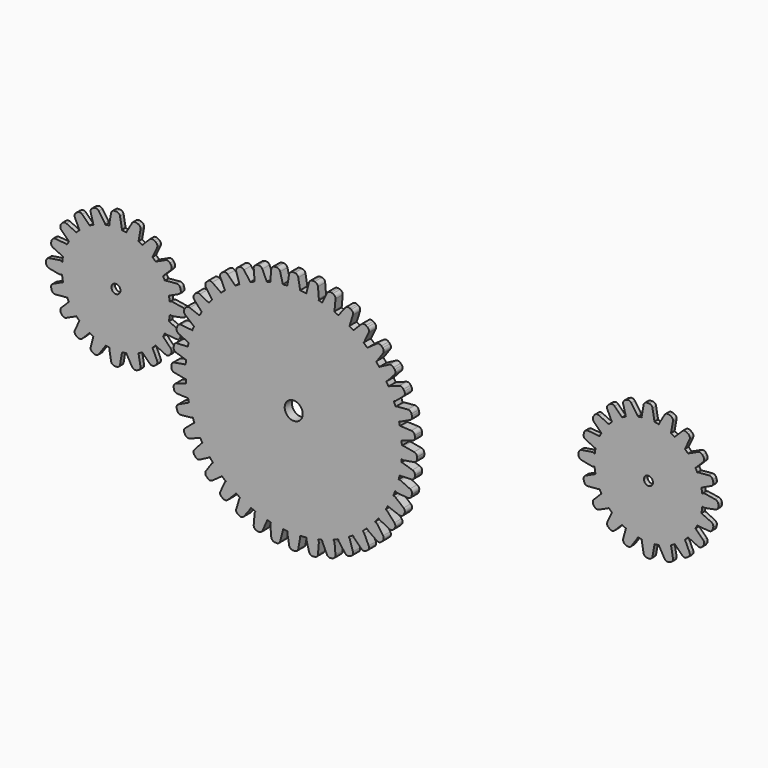
from build123d import *

# Parameters (mm, degrees)
F1_DEPTH = 6.35
F0_R     = 12.7
F2_DEPTH = 12.7
F0_R_2   = 6.35
F3_DEPTH = 6.35


# Not quite as in the source:
# - a feature names something its author has since deleted; it is built from what else it names


with BuildPart() as f1:
    # F0 (on Front) → F1 (new body)
    with BuildSketch(Plane.XZ):
        with BuildLine():
            ThreePointArc((569.0594632966, 55.4081884367), (569.8879744655, 59.9600322896), (570.4387118167, 64.5537673263))
            ThreePointArc((570.4387118167, 64.5537673263), (568.9804312729, 66.3079527176), (568.4367834806, 68.5233975057))
            Line((568.4367834806, 68.5233975057), (568.3970793336, 71.3232904673))
            Line((568.3970793336, 71.3232904673), (500.8900059223, 71.3232904673))
            ThreePointArc((500.8900059223, 71.3232904673), (499.0301339829, 66.8331624067), (494.5400059223, 64.9732904673))
            Line((494.5400059223, 64.9732904673), (494.5400059223, -0.3120452166))
            Line((494.5400059223, -0.3120452166), (497.7978995991, -0.3120452166))
            ThreePointArc((497.7978995991, -0.3120452166), (501.0317339111, -1.4743015238), (502.7858263626, -4.4292437825))
            ThreePointArc((502.7858263626, -4.4292437825), (506.0662797675, -3.9999132036), (509.3250050347, -3.4285911227))
            ThreePointArc((509.3250050348, -3.4285911227), (509.9976617201, -0.1002598118), (512.6168727875, 2.0607560873))
            Line((512.6168727875, 2.0607560873), (519.7773305579, 4.6669495794))
            ThreePointArc((519.7773305579, 4.6669495794), (523.4863017797, 4.5751432587), (526.1436883273, 1.9860907946))
            ThreePointArc((526.1436883273, 1.9860907946), (528.912144359, 3.3159666022), (531.6247607403, 4.7563244849))
            ThreePointArc((531.6247607403, 4.7563244849), (530.2946375644, 8.7497147606), (532.4325561523, 12.3754143715))
            Line((532.4325561523, 12.3754143715), (538.6744947298, 16.7460668165))
            ThreePointArc((538.6744947298, 16.7460668165), (542.6920561228, 17.5434073883), (545.9920497123, 15.1171770112))
            ThreePointArc((545.9920497123, 15.1171770112), (548.2003085288, 17.2214242871), (550.3225818533, 19.4123646183))
            ThreePointArc((550.3225818533, 19.4123646183), (548.1921358653, 22.6958576232), (549.0286946297, 26.5195071697))
            Line((549.0286946297, 26.5195071697), (553.3993470747, 32.7614457472))
            ThreePointArc((553.3993470747, 32.7614457472), (556.8977046725, 34.8842355479), (560.8262141804, 33.7390039266))
            ThreePointArc((560.8262141804, 33.7390039266), (562.1419162355, 36.1605015847), (563.3691961646, 38.6279915607))
            ThreePointArc((563.3691961646, 38.6279915607), (560.9829608467, 41.0874359569), (560.7014894485, 44.5026606321))
            Line((560.7014894485, 44.5026606321), (562.6736905722, 51.8630154285))
            ThreePointArc((562.6736905722, 51.8630154285), (565.1148450748, 54.9896652727), (569.0594632966, 55.4081884367))
        make_face()
        with BuildLine():
            ThreePointArc((488.1900059223, 71.3232904673), (490.0498778618, 75.8134185278), (494.5400059223, 77.6732904673))
            Line((494.5400059223, 77.6732904673), (494.5400059223, 142.9586261511))
            Line((494.5400059223, 142.9586261511), (490.1778995991, 142.9586261511))
            ThreePointArc((490.1778995991, 142.9586261511), (486.9936006991, 144.0805154256), (485.2157706112, 146.9506574442))
            ThreePointArc((485.2157706112, 146.9506574442), (482.3975220212, 146.5496162097), (479.5962192549, 146.0435905204))
            ThreePointArc((479.5962192549, 146.0435905204), (479.0648250211, 142.8630265455), (476.7259389086, 140.6431214162))
            Line((476.7259389086, 140.6431214162), (469.8198735714, 137.4227702618))
            ThreePointArc((469.8198735714, 137.4227702618), (465.5801709332, 137.3979283883), (462.7982295208, 140.5973810847))
            ThreePointArc((462.7982295208, 140.5973810847), (460.100131055, 139.2963367365), (457.4552511044, 137.8902564496))
            ThreePointArc((457.4552511044, 137.8902564496), (458.7853742803, 133.8968661739), (456.6474556923, 130.271166563))
            Line((456.6474556923, 130.271166563), (450.4055171148, 125.900514118))
            ThreePointArc((450.4055171148, 125.900514118), (446.3879557219, 125.1031735462), (443.0879621323, 127.5294039233))
            ThreePointArc((443.0879621323, 127.5294039233), (440.8797033158, 125.4251566474), (438.7574299913, 123.2342163163))
            ThreePointArc((438.7574299913, 123.2342163163), (440.8878759793, 119.9507233114), (440.051317215, 116.1270737648))
            Line((440.051317215, 116.1270737648), (435.68066477, 109.8851351873))
            ThreePointArc((435.68066477, 109.8851351873), (432.1823071722, 107.7623453866), (428.2537976643, 108.9075770079))
            ThreePointArc((428.2537976643, 108.9075770079), (426.9380956091, 106.4860793499), (425.71081568, 104.0185893739))
            ThreePointArc((425.71081568, 104.0185893739), (428.0970509979, 101.5591449776), (428.3785223961, 98.1439203024))
            Line((428.3785223961, 98.1439203024), (426.4063212724, 90.7835655061))
            ThreePointArc((426.4063212724, 90.7835655061), (423.9651667698, 87.6569156618), (420.020548548, 87.2383924978))
            ThreePointArc((420.020548548, 87.2383924978), (419.3550648664, 83.7194446457), (418.8556574238, 80.173114892))
            ThreePointArc((418.8556574238, 80.173114892), (420.2687386114, 78.3767003311), (420.751273632, 76.1426314712))
            Line((420.751273632, 76.1426314712), (420.682932511, 71.3232904673))
            Line((420.682932511, 71.3232904673), (488.1900059223, 71.3232904673))
        make_face()
        with BuildLine():
            Line((494.5400059223, -0.3120452166), (494.5400059223, 64.9732904673))
            ThreePointArc((494.5400059223, 64.9732904673), (490.0498778618, 66.8331624067), (488.1900059223, 71.3232904673))
            Line((488.1900059223, 71.3232904673), (420.682932511, 71.3232904673))
            Line((420.682932511, 71.3232904673), (420.643228364, 68.5233975057))
            ThreePointArc((420.643228364, 68.5233975057), (420.0995805717, 66.3079527176), (418.6413000279, 64.5537673263))
            ThreePointArc((418.6413000279, 64.5537673263), (419.1920373791, 59.9600322896), (420.020548548, 55.4081884367))
            ThreePointArc((420.020548548, 55.4081884367), (423.9651667698, 54.9896652727), (426.4063212724, 51.8630154285))
            Line((426.4063212724, 51.8630154285), (428.3785223961, 44.5026606321))
            ThreePointArc((428.3785223961, 44.5026606321), (428.0970509979, 41.0874359569), (425.71081568, 38.6279915607))
            ThreePointArc((425.71081568, 38.6279915607), (426.9380956091, 36.1605015847), (428.2537976643, 33.7390039266))
            ThreePointArc((428.2537976643, 33.7390039266), (432.1823071722, 34.8842355479), (435.68066477, 32.7614457472))
            Line((435.68066477, 32.7614457472), (440.051317215, 26.5195071697))
            ThreePointArc((440.051317215, 26.5195071697), (440.8878759793, 22.6958576232), (438.7574299913, 19.4123646183))
            ThreePointArc((438.7574299913, 19.4123646183), (440.8797033158, 17.2214242871), (443.0879621323, 15.1171770112))
            ThreePointArc((443.0879621323, 15.1171770112), (446.3879557219, 17.5434073883), (450.4055171148, 16.7460668165))
            Line((450.4055171148, 16.7460668165), (456.6474556923, 12.3754143715))
            ThreePointArc((456.6474556923, 12.3754143715), (458.7853742803, 8.7497147606), (457.4552511044, 4.7563244849))
            ThreePointArc((457.4552511044, 4.7563244849), (460.100131055, 3.350244198), (462.7982295208, 2.0491998498))
            ThreePointArc((462.7982295208, 2.0491998498), (465.5801709332, 5.2486525462), (469.8198735714, 5.2238106728))
            Line((469.8198735714, 5.2238106728), (476.7259389086, 2.0034595183))
            ThreePointArc((476.7259389086, 2.0034595183), (479.0648250211, -0.216445611), (479.5962192549, -3.3970095859))
            ThreePointArc((479.5962192549, -3.3970095859), (482.3975220212, -3.9030352752), (485.2157706112, -4.3040765097))
            ThreePointArc((485.2157706112, -4.3040765097), (486.9936006991, -1.433934491), (490.1778995991, -0.3120452166))
            Line((490.1778995991, -0.3120452166), (494.5400059223, -0.3120452166))
        make_face()
        with BuildLine():
            ThreePointArc((568.3287382126, 76.1426314712), (568.8112732333, 78.3767003311), (570.2243544209, 80.173114892))
            ThreePointArc((570.2243544209, 80.173114892), (569.7249469782, 83.7194446457), (569.0594632966, 87.2383924978))
            ThreePointArc((569.0594632966, 87.2383924978), (565.1148450748, 87.6569156618), (562.6736905722, 90.7835655061))
            Line((562.6736905722, 90.7835655061), (560.7014894485, 98.1439203024))
            ThreePointArc((560.7014894485, 98.1439203024), (560.9829608467, 101.5591449776), (563.3691961646, 104.0185893739))
            ThreePointArc((563.3691961646, 104.0185893739), (562.1419162355, 106.4860793499), (560.8262141804, 108.9075770079))
            ThreePointArc((560.8262141804, 108.9075770079), (556.8977046725, 107.7623453866), (553.3993470747, 109.8851351873))
            Line((553.3993470747, 109.8851351873), (549.0286946297, 116.1270737648))
            ThreePointArc((549.0286946297, 116.1270737648), (548.1921358653, 119.9507233114), (550.3225818533, 123.2342163163))
            ThreePointArc((550.3225818533, 123.2342163163), (548.2003085288, 125.4251566474), (545.9920497123, 127.5294039233))
            ThreePointArc((545.9920497123, 127.5294039233), (542.6920561228, 125.1031735462), (538.6744947298, 125.900514118))
            Line((538.6744947298, 125.900514118), (532.4325561523, 130.271166563))
            ThreePointArc((532.4325561523, 130.271166563), (530.2946375644, 133.8968661739), (531.6247607403, 137.8902564496))
            ThreePointArc((531.6247607403, 137.8902564496), (528.912144359, 139.3306143324), (526.1436883273, 140.6604901399))
            ThreePointArc((526.1436883273, 140.6604901399), (523.4863017797, 138.0714376758), (519.7773305579, 137.9796313551))
            Line((519.7773305579, 137.9796313551), (512.6168727875, 140.5858248472))
            ThreePointArc((512.6168727875, 140.5858248472), (509.9976617201, 142.7468407464), (509.3250050348, 146.0751720573))
            ThreePointArc((509.3250050347, 146.0751720573), (506.0662797675, 146.6464941381), (502.7858263626, 147.0758247171))
            ThreePointArc((502.7858263626, 147.0758247171), (501.0317339111, 144.1208824583), (497.7978995991, 142.9586261511))
            Line((497.7978995991, 142.9586261511), (494.5400059223, 142.9586261511))
            Line((494.5400059223, 142.9586261511), (494.5400059223, 77.6732904673))
            ThreePointArc((494.5400059223, 77.6732904673), (499.0301339829, 75.8134185278), (500.8900059223, 71.3232904673))
            Line((500.8900059223, 71.3232904673), (568.3970793336, 71.3232904673))
            Line((568.3970793336, 71.3232904673), (568.3287382126, 76.1426314712))
        make_face()
        with BuildLine():
            ThreePointArc((462.7982295208, 140.5973810847), (471.0389261796, 143.8087321154), (479.5962192549, 146.0435905204))
            ThreePointArc((479.5962192549, 146.0435905204), (479.2888023616, 147.1509824466), (478.740330524, 148.160933271))
            Line((478.740330524, 148.160933271), (470.3504690932, 160.1428971502))
            ThreePointArc((470.3504690932, 160.1428971502), (467.5039774573, 162.1360320511), (464.0422759386, 161.8331724117))
            Line((464.0422759386, 161.8331724117), (461.7402541595, 160.7597220269))
            ThreePointArc((461.7402541595, 160.7597220269), (459.283111371, 158.3025792384), (458.9802517316, 154.8408777196))
            Line((458.9802517316, 154.8408777196), (462.7660696042, 140.7120130708))
            ThreePointArc((462.7660696042, 140.7120130708), (462.7818137284, 140.6546028598), (462.7982295208, 140.5973810847))
        make_face()
        with BuildLine():
            ThreePointArc((569.7274945394, 55.1522582375), (569.3979896065, 55.2919971757), (569.0594632966, 55.4081884367))
            ThreePointArc((569.0594632966, 55.4081884367), (566.7037256517, 46.8521328562), (563.3691961646, 38.6279915607))
            ThreePointArc((563.3691961646, 38.6279915607), (564.2442404728, 38.2944470813), (565.1656414729, 38.1271908167))
            Line((565.1656414729, 38.1271908167), (579.7372572949, 36.852339623))
            ThreePointArc((579.7372572949, 36.852339623), (583.0937767648, 37.7517163043), (585.0869116656, 40.5982079402))
            Line((585.0869116656, 40.5982079402), (585.7443120402, 43.051659539))
            ThreePointArc((585.7443120402, 43.051659539), (585.4414524008, 46.5133610577), (582.9843096123, 48.9705038463))
            Line((582.9843096123, 48.9705038463), (569.7274945394, 55.1522582375))
        make_face()
        with BuildLine():
            Line((396.1161720733, 71.3232904673), (418.3400059223, 71.3232904673))
            ThreePointArc((418.3400059223, 71.3232904673), (418.469028028, 75.7557076639), (418.8556574238, 80.173114892))
            ThreePointArc((418.8556574238, 80.173114892), (416.9704318638, 81.1258646147), (414.860676138, 81.2294900132))
            Line((414.860676138, 81.2294900132), (400.4210533594, 78.8939970795))
            ThreePointArc((400.4210533594, 78.8939970795), (397.3873470896, 77.1993798265), (396.1526722329, 73.9511988949))
            Line((396.1526722329, 73.9511988949), (396.1166571436, 71.4114542397))
            ThreePointArc((396.1166571436, 71.4114542397), (396.1162233409, 71.3673734058), (396.1161720733, 71.3232904673))
        make_face()
        with BuildLine():
            ThreePointArc((570.2243544209, 80.173114892), (570.6109838166, 75.7557076639), (570.7400059223, 71.3232904673))
            ThreePointArc((570.7400059223, 71.3232904673), (570.6646451305, 67.9351780985), (570.4387118167, 64.5537673263))
            ThreePointArc((570.4387118167, 64.5537673263), (572.3529975508, 63.6504109286), (574.4692527316, 63.6056151396))
            Line((574.4692527316, 63.6056151396), (588.8368453314, 66.3496115162))
            ThreePointArc((588.8368453314, 66.3496115162), (591.8212800572, 68.1295695869), (592.9633547011, 71.4114542397))
            Line((592.9633547011, 71.4114542397), (592.9273396117, 73.9511988949))
            ThreePointArc((592.9273396117, 73.9511988949), (591.6926647551, 77.1993798265), (588.6589584852, 78.8939970795))
            Line((588.6589584852, 78.8939970795), (574.2193357067, 81.2294900132))
            ThreePointArc((574.2193357067, 81.2294900132), (572.1095799808, 81.1258646147), (570.2243544209, 80.173114892))
        make_face()
        with BuildLine():
            ThreePointArc((457.3257898441, 4.6220195381), (457.3911370015, 4.6885777192), (457.4552511044, 4.7563244849))
            ThreePointArc((457.4552511044, 4.7563244849), (449.9695224921, 9.5178537582), (443.0879621323, 15.1171770112))
            ThreePointArc((443.0879621323, 15.1171770112), (442.9837110701, 14.9265676894), (442.88770526, 14.7316752011))
            Line((442.88770526, 14.7316752011), (436.7059508688, 1.4748601283))
            ThreePointArc((436.7059508688, 1.4748601283), (436.4030912294, -1.9868413905), (438.3962261303, -4.8333330264))
            Line((438.3962261303, -4.8333330264), (440.4768723227, -6.2902171747))
            ThreePointArc((440.4768723227, -6.2902171747), (443.8333917926, -7.189593856), (446.9827430678, -5.7210272381))
            Line((446.9827430678, -5.7210272381), (457.3257898441, 4.6220195381))
        make_face()
        with BuildLine():
            ThreePointArc((526.1436883273, 1.9860907946), (517.8918182352, -1.210376624), (509.3250050347, -3.4285911227))
            ThreePointArc((509.3250050348, -3.4285911227), (509.5525344018, -4.370926426), (509.9549260643, -5.2528824263))
            Line((509.9549260643, -5.2528824263), (517.2685645779, -17.92047592))
            ThreePointArc((517.2685645779, -17.92047592), (519.9305113011, -20.1541144336), (523.4054359573, -20.1541144336))
            Line((523.4054359573, -20.1541144336), (525.7922552141, -19.2853832696))
            ThreePointArc((525.7922552141, -19.2853832696), (528.4542019372, -17.051744756), (529.0576162713, -13.6296120134))
            Line((529.0576162713, -13.6296120134), (526.5176162713, 0.7754438084))
            ThreePointArc((526.5176162713, 0.7754438084), (526.3685459102, 1.3924713574), (526.1436883273, 1.9860907946))
        make_face()
        with BuildLine():
            ThreePointArc((561.1527419081, 33.439779899), (560.9927405353, 33.5929521009), (560.8262141804, 33.7390039266))
            ThreePointArc((560.8262141804, 33.7390039266), (555.993322894, 26.2685478403), (550.3225818533, 19.4123646183))
            ThreePointArc((550.3225818533, 19.4123646183), (550.6744396962, 19.1923023788), (551.043086245, 19.0016953149))
            Line((551.043086245, 19.0016953149), (564.2999013179, 12.8199409237))
            ThreePointArc((564.2999013179, 12.8199409237), (567.7616028367, 12.5170812843), (570.6080944725, 14.5102161852))
            Line((570.6080944725, 14.5102161852), (572.0649786209, 16.5908623777))
            ThreePointArc((572.0649786209, 16.5908623777), (572.9643553022, 19.9473818475), (571.4957886843, 23.0967331228))
            Line((571.4957886843, 23.0967331228), (561.1527419081, 33.439779899))
        make_face()
        with BuildLine():
            ThreePointArc((546.1923065846, 14.7316752011), (546.0963007745, 14.9265676894), (545.9920497123, 15.1171770112))
            ThreePointArc((545.9920497123, 15.1171770112), (539.1104893525, 9.5178537582), (531.6247607403, 4.7563244849))
            ThreePointArc((531.6247607403, 4.7563244849), (531.6888748432, 4.6885777192), (531.7542220006, 4.6220195381))
            Line((531.7542220006, 4.6220195381), (542.0972687768, -5.7210272381))
            ThreePointArc((542.0972687768, -5.7210272381), (545.2466200521, -7.189593856), (548.6031395219, -6.2902171747))
            Line((548.6031395219, -6.2902171747), (550.6837857144, -4.8333330264))
            ThreePointArc((550.6837857144, -4.8333330264), (552.6769206153, -1.9868413905), (552.3740609759, 1.4748601283))
            Line((552.3740609759, 1.4748601283), (546.1923065846, 14.7316752011))
        make_face()
        with BuildLine():
            ThreePointArc((478.740330524, -5.5143523365), (479.2888023616, -4.5044015121), (479.5962192549, -3.3970095859))
            ThreePointArc((479.5962192549, -3.3970095859), (471.0389261796, -1.1621511809), (462.7982295208, 2.0491998498))
            ThreePointArc((462.7982295208, 2.0491998498), (462.7818137284, 1.9919780748), (462.7660696042, 1.9345678637))
            Line((462.7660696042, 1.9345678637), (458.9802517316, -12.1942967851))
            ThreePointArc((458.9802517316, -12.1942967851), (459.283111371, -15.6559983039), (461.7402541595, -18.1131410924))
            Line((461.7402541595, -18.1131410924), (464.0422759386, -19.1865914772))
            ThreePointArc((464.0422759386, -19.1865914772), (467.5039774573, -19.4894511166), (470.3504690932, -17.4963162157))
            Line((470.3504690932, -17.4963162157), (478.740330524, -5.5143523365))
        make_face()
        with BuildLine():
            ThreePointArc((550.3225818533, 123.2342163163), (555.993322894, 116.3780330942), (560.8262141804, 108.9075770079))
            ThreePointArc((560.8262141804, 108.9075770079), (560.9927405353, 109.0536288337), (561.1527419081, 109.2068010356))
            Line((561.1527419081, 109.2068010356), (571.4957886843, 119.5498478118))
            ThreePointArc((571.4957886843, 119.5498478118), (572.9643553022, 122.699199087), (572.0649786209, 126.0557185569))
            Line((572.0649786209, 126.0557185569), (570.6080944725, 128.1363647494))
            ThreePointArc((570.6080944725, 128.1363647494), (567.7616028367, 130.1294996502), (564.2999013179, 129.8266400108))
            Line((564.2999013179, 129.8266400108), (551.043086245, 123.6448856196))
            ThreePointArc((551.043086245, 123.6448856196), (550.6744396962, 123.4542785557), (550.3225818533, 123.2342163163))
        make_face()
        with BuildLine():
            ThreePointArc((438.7574299913, 19.4123646183), (433.0866889507, 26.2685478403), (428.2537976643, 33.7390039266))
            ThreePointArc((428.2537976643, 33.7390039266), (428.0872713093, 33.5929521009), (427.9272699366, 33.439779899))
            Line((427.9272699366, 33.439779899), (417.5842231603, 23.0967331228))
            ThreePointArc((417.5842231603, 23.0967331228), (416.1156565425, 19.9473818475), (417.0150332238, 16.5908623777))
            Line((417.0150332238, 16.5908623777), (418.4719173721, 14.5102161852))
            ThreePointArc((418.4719173721, 14.5102161852), (421.318409008, 12.5170812843), (424.7801105267, 12.8199409237))
            Line((424.7801105267, 12.8199409237), (438.0369255996, 19.0016953149))
            ThreePointArc((438.0369255996, 19.0016953149), (438.4055721485, 19.1923023788), (438.7574299913, 19.4123646183))
        make_face()
        with BuildLine():
            Line((494.5400059223, -24.8771010384), (494.5400059223, -4.8767095327))
            ThreePointArc((494.5400059223, -4.8767095327), (489.8691047053, -4.7334165468), (485.2157706112, -4.3040765097))
            ThreePointArc((485.2157706112, -4.3040765097), (485.0989829941, -5.287135162), (485.1750762138, -6.2741779591))
            Line((485.1750762138, -6.2741779591), (487.7150762138, -20.6792337809))
            ThreePointArc((487.7150762138, -20.6792337809), (489.4525385419, -23.6886068094), (492.7178995991, -24.8771010384))
            Line((492.7178995991, -24.8771010384), (494.5400059223, -24.8771010384))
        make_face()
        with BuildLine():
            ThreePointArc((553.3993470747, 109.8851351873), (556.8977046725, 107.7623453866), (560.8262141804, 108.9075770079))
            ThreePointArc((560.8262141804, 108.9075770079), (555.993322894, 116.3780330942), (550.3225818533, 123.2342163163))
            ThreePointArc((550.3225818533, 123.2342163163), (548.1921358653, 119.9507233114), (549.0286946297, 116.1270737648))
            Line((549.0286946297, 116.1270737648), (553.3993470747, 109.8851351873))
        make_face()
        with BuildLine():
            ThreePointArc((512.6168727875, 2.0607560873), (509.9976617201, -0.1002598118), (509.3250050348, -3.4285911227))
            ThreePointArc((509.3250050347, -3.4285911227), (517.8918182352, -1.210376624), (526.1436883273, 1.9860907946))
            ThreePointArc((526.1436883273, 1.9860907946), (523.4863017797, 4.5751432587), (519.7773305579, 4.6669495794))
            Line((519.7773305579, 4.6669495794), (512.6168727875, 2.0607560873))
        make_face()
        with BuildLine():
            ThreePointArc((456.6474556923, 130.271166563), (458.7853742803, 133.8968661739), (457.4552511044, 137.8902564496))
            ThreePointArc((457.4552511044, 137.8902564496), (449.9695224921, 133.1287271763), (443.0879621323, 127.5294039233))
            ThreePointArc((443.0879621323, 127.5294039233), (446.3879557219, 125.1031735462), (450.4055171148, 125.900514118))
            Line((450.4055171148, 125.900514118), (456.6474556923, 130.271166563))
        make_face()
        with BuildLine():
            ThreePointArc((509.9549260643, 147.8994633608), (509.5525344018, 147.0175073605), (509.3250050348, 146.0751720573))
            ThreePointArc((509.3250050347, 146.0751720573), (517.8918182352, 143.8569575585), (526.1436883273, 140.6604901399))
            ThreePointArc((526.1436883273, 140.6604901399), (526.3685459102, 141.2541095771), (526.5176162713, 141.8711371261))
            Line((526.5176162713, 141.8711371261), (529.0576162713, 156.276192948))
            ThreePointArc((529.0576162713, 156.276192948), (528.4542019372, 159.6983256905), (525.7922552141, 161.9319642041))
            Line((525.7922552141, 161.9319642041), (523.4054359573, 162.8006953681))
            ThreePointArc((523.4054359573, 162.8006953681), (519.9305113011, 162.8006953681), (517.2685645779, 160.5670568545))
            Line((517.2685645779, 160.5670568545), (509.9549260643, 147.8994633608))
        make_face()
        with BuildLine():
            ThreePointArc((502.7858263626, -4.4292437825), (498.6689821977, -4.7647608609), (494.5400059223, -4.8767095327))
            Line((494.5400059223, -4.8767095327), (494.5400059223, -24.8771010384))
            Line((494.5400059223, -24.8771010384), (495.2578995991, -24.8771010384))
            ThreePointArc((495.2578995991, -24.8771010384), (498.5232606563, -23.6886068094), (500.2607229844, -20.6792337809))
            Line((500.2607229844, -20.6792337809), (502.8007229844, -6.2741779591))
            ThreePointArc((502.8007229844, -6.2741779591), (502.877734012, -5.3510289176), (502.7858263626, -4.4292437825))
        make_face()
        with BuildLine():
            ThreePointArc((419.3525173052, 87.494322697), (419.6820222381, 87.3545837588), (420.020548548, 87.2383924978))
            ThreePointArc((420.020548548, 87.2383924978), (422.376286193, 95.7944480783), (425.71081568, 104.0185893739))
            ThreePointArc((425.71081568, 104.0185893739), (424.8357713718, 104.3521338532), (423.9143703717, 104.5193901178))
            Line((423.9143703717, 104.5193901178), (409.3427545497, 105.7942413115))
            ThreePointArc((409.3427545497, 105.7942413115), (405.9862350799, 104.8948646302), (403.993100179, 102.0483729943))
            Line((403.993100179, 102.0483729943), (403.3356998044, 99.5949213955))
            ThreePointArc((403.3356998044, 99.5949213955), (403.6385594438, 96.1332198768), (406.0957022323, 93.6760770883))
            Line((406.0957022323, 93.6760770883), (419.3525173052, 87.494322697))
        make_face()
        with BuildLine():
            ThreePointArc((438.7574299913, 123.2342163163), (433.0866889507, 116.3780330942), (428.2537976643, 108.9075770079))
            ThreePointArc((428.2537976643, 108.9075770079), (432.1823071722, 107.7623453866), (435.68066477, 109.8851351873))
            Line((435.68066477, 109.8851351873), (440.051317215, 116.1270737648))
            ThreePointArc((440.051317215, 116.1270737648), (440.8878759793, 119.9507233114), (438.7574299913, 123.2342163163))
        make_face()
        with BuildLine():
            ThreePointArc((538.6744947298, 125.900514118), (542.6920561228, 125.1031735462), (545.9920497123, 127.5294039233))
            ThreePointArc((545.9920497123, 127.5294039233), (539.1104893525, 133.1287271763), (531.6247607403, 137.8902564496))
            ThreePointArc((531.6247607403, 137.8902564496), (530.2946375644, 133.8968661739), (532.4325561523, 130.271166563))
            Line((532.4325561523, 130.271166563), (538.6744947298, 125.900514118))
        make_face()
        with BuildLine():
            ThreePointArc((550.3225818533, 19.4123646183), (555.993322894, 26.2685478403), (560.8262141804, 33.7390039266))
            ThreePointArc((560.8262141804, 33.7390039266), (556.8977046725, 34.8842355479), (553.3993470747, 32.7614457472))
            Line((553.3993470747, 32.7614457472), (549.0286946297, 26.5195071697))
            ThreePointArc((549.0286946297, 26.5195071697), (548.1921358653, 22.6958576232), (550.3225818533, 19.4123646183))
        make_face()
        with BuildLine():
            ThreePointArc((563.3691961646, 104.0185893739), (566.7037256517, 95.7944480783), (569.0594632966, 87.2383924978))
            ThreePointArc((569.0594632966, 87.2383924978), (569.3979896065, 87.3545837588), (569.7274945394, 87.494322697))
            Line((569.7274945394, 87.494322697), (582.9843096123, 93.6760770883))
            ThreePointArc((582.9843096123, 93.6760770883), (585.4414524008, 96.1332198768), (585.7443120402, 99.5949213955))
            Line((585.7443120402, 99.5949213955), (585.0869116656, 102.0483729943))
            ThreePointArc((585.0869116656, 102.0483729943), (583.0937767648, 104.8948646302), (579.7372572949, 105.7942413115))
            Line((579.7372572949, 105.7942413115), (565.1656414729, 104.5193901178))
            ThreePointArc((565.1656414729, 104.5193901178), (564.2442404728, 104.3521338532), (563.3691961646, 104.0185893739))
        make_face()
        with BuildLine():
            Line((494.5400059223, 167.5236819729), (494.5400059223, 147.5232904673))
            ThreePointArc((494.5400059223, 147.5232904673), (498.6689821977, 147.4113417954), (502.7858263626, 147.0758247171))
            ThreePointArc((502.7858263626, 147.0758247171), (502.877734012, 147.9976098521), (502.8007229844, 148.9207588936))
            Line((502.8007229844, 148.9207588936), (500.2607229844, 163.3258147155))
            ThreePointArc((500.2607229844, 163.3258147155), (498.5232606563, 166.335187744), (495.2578995991, 167.5236819729))
            Line((495.2578995991, 167.5236819729), (494.5400059223, 167.5236819729))
        make_face()
        with BuildLine():
            ThreePointArc((418.6413000279, 64.5537673263), (418.4153667141, 67.9351780985), (418.3400059223, 71.3232904673))
            Line((418.3400059223, 71.3232904673), (396.1161720733, 71.3232904673))
            ThreePointArc((396.1161720733, 71.3232904673), (397.2867340891, 68.0955228661), (400.2431665132, 66.3496115162))
            Line((400.2431665132, 66.3496115162), (414.6107591131, 63.6056151396))
            ThreePointArc((414.6107591131, 63.6056151396), (416.7270142939, 63.6504109286), (418.6413000279, 64.5537673263))
        make_face()
        with BuildLine():
            ThreePointArc((427.9272699366, 109.2068010356), (428.0872713093, 109.0536288337), (428.2537976643, 108.9075770079))
            ThreePointArc((428.2537976643, 108.9075770079), (433.0866889507, 116.3780330942), (438.7574299913, 123.2342163163))
            ThreePointArc((438.7574299913, 123.2342163163), (438.4055721485, 123.4542785557), (438.0369255996, 123.6448856196))
            Line((438.0369255996, 123.6448856196), (424.7801105267, 129.8266400108))
            ThreePointArc((424.7801105267, 129.8266400108), (421.318409008, 130.1294996502), (418.4719173721, 128.1363647494))
            Line((418.4719173721, 128.1363647494), (417.0150332238, 126.0557185569))
            ThreePointArc((417.0150332238, 126.0557185569), (416.1156565425, 122.699199087), (417.5842231603, 119.5498478118))
            Line((417.5842231603, 119.5498478118), (427.9272699366, 109.2068010356))
        make_face()
        with BuildLine():
            ThreePointArc((425.71081568, 104.0185893739), (422.376286193, 95.7944480783), (420.020548548, 87.2383924978))
            ThreePointArc((420.020548548, 87.2383924978), (423.9651667698, 87.6569156618), (426.4063212724, 90.7835655061))
            Line((426.4063212724, 90.7835655061), (428.3785223961, 98.1439203024))
            ThreePointArc((428.3785223961, 98.1439203024), (428.0970509979, 101.5591449776), (425.71081568, 104.0185893739))
        make_face()
        with BuildLine():
            ThreePointArc((425.71081568, 38.6279915607), (422.376286193, 46.8521328562), (420.020548548, 55.4081884367))
            ThreePointArc((420.020548548, 55.4081884367), (419.6820222381, 55.2919971757), (419.3525173052, 55.1522582375))
            Line((419.3525173052, 55.1522582375), (406.0957022323, 48.9705038463))
            ThreePointArc((406.0957022323, 48.9705038463), (403.6385594438, 46.5133610577), (403.3356998044, 43.051659539))
            Line((403.3356998044, 43.051659539), (403.993100179, 40.5982079402))
            ThreePointArc((403.993100179, 40.5982079402), (405.9862350799, 37.7517163043), (409.3427545497, 36.852339623))
            Line((409.3427545497, 36.852339623), (423.9143703717, 38.1271908167))
            ThreePointArc((423.9143703717, 38.1271908167), (424.8357713718, 38.2944470813), (425.71081568, 38.6279915607))
        make_face()
        with BuildLine():
            ThreePointArc((435.68066477, 32.7614457472), (432.1823071722, 34.8842355479), (428.2537976643, 33.7390039266))
            ThreePointArc((428.2537976643, 33.7390039266), (433.0866889507, 26.2685478403), (438.7574299913, 19.4123646183))
            ThreePointArc((438.7574299913, 19.4123646183), (440.8878759793, 22.6958576232), (440.051317215, 26.5195071697))
            Line((440.051317215, 26.5195071697), (435.68066477, 32.7614457472))
        make_face()
        with BuildLine():
            ThreePointArc((443.0879621323, 127.5294039233), (449.9695224921, 133.1287271763), (457.4552511044, 137.8902564496))
            ThreePointArc((457.4552511044, 137.8902564496), (457.3911370015, 137.9580032153), (457.3257898441, 138.0245613964))
            Line((457.3257898441, 138.0245613964), (446.9827430678, 148.3676081727))
            ThreePointArc((446.9827430678, 148.3676081727), (443.8333917926, 149.8361747905), (440.4768723227, 148.9367981092))
            Line((440.4768723227, 148.9367981092), (438.3962261303, 147.4799139609))
            ThreePointArc((438.3962261303, 147.4799139609), (436.4030912294, 144.633422325), (436.7059508688, 141.1717208063))
            Line((436.7059508688, 141.1717208063), (442.88770526, 127.9149057334))
            ThreePointArc((442.88770526, 127.9149057334), (442.9837110701, 127.7200132452), (443.0879621323, 127.5294039233))
        make_face()
        with BuildLine():
            ThreePointArc((476.7259389086, 140.6431214162), (479.0648250211, 142.8630265455), (479.5962192549, 146.0435905204))
            ThreePointArc((479.5962192549, 146.0435905204), (471.0389261796, 143.8087321154), (462.7982295208, 140.5973810847))
            ThreePointArc((462.7982295208, 140.5973810847), (465.5801709332, 137.3979283883), (469.8198735714, 137.4227702618))
            Line((469.8198735714, 137.4227702618), (476.7259389086, 140.6431214162))
        make_face()
        with BuildLine():
            ThreePointArc((485.2157706112, 146.9506574442), (489.8691047053, 147.3799974813), (494.5400059223, 147.5232904673))
            Line((494.5400059223, 147.5232904673), (494.5400059223, 167.5236819729))
            Line((494.5400059223, 167.5236819729), (492.7178995991, 167.5236819729))
            ThreePointArc((492.7178995991, 167.5236819729), (489.4525385419, 166.335187744), (487.7150762138, 163.3258147155))
            Line((487.7150762138, 163.3258147155), (485.1750762138, 148.9207588936))
            ThreePointArc((485.1750762138, 148.9207588936), (485.0989829941, 147.9337160965), (485.2157706112, 146.9506574442))
        make_face()
        with BuildLine():
            ThreePointArc((443.0879621323, 15.1171770112), (449.9695224921, 9.5178537582), (457.4552511044, 4.7563244849))
            ThreePointArc((457.4552511044, 4.7563244849), (458.7853742803, 8.7497147606), (456.6474556923, 12.3754143715))
            Line((456.6474556923, 12.3754143715), (450.4055171148, 16.7460668165))
            ThreePointArc((450.4055171148, 16.7460668165), (446.3879557219, 17.5434073883), (443.0879621323, 15.1171770112))
        make_face()
        with BuildLine():
            ThreePointArc((531.6247607403, 4.7563244849), (539.1104893525, 9.5178537582), (545.9920497123, 15.1171770112))
            ThreePointArc((545.9920497123, 15.1171770112), (542.6920561228, 17.5434073883), (538.6744947298, 16.7460668165))
            Line((538.6744947298, 16.7460668165), (532.4325561523, 12.3754143715))
            ThreePointArc((532.4325561523, 12.3754143715), (530.2946375644, 8.7497147606), (531.6247607403, 4.7563244849))
        make_face()
        with BuildLine():
            Line((497.7978995991, -0.3120452166), (494.5400059223, -0.3120452166))
            Line((494.5400059223, -0.3120452166), (494.5400059223, -4.8767095327))
            ThreePointArc((494.5400059223, -4.8767095327), (498.6689821977, -4.7647608609), (502.7858263626, -4.4292437825))
            ThreePointArc((502.7858263626, -4.4292437825), (501.0317339111, -1.4743015238), (497.7978995991, -0.3120452166))
        make_face()
        with BuildLine():
            ThreePointArc((531.6247607403, 137.8902564496), (539.1104893525, 133.1287271763), (545.9920497123, 127.5294039233))
            ThreePointArc((545.9920497123, 127.5294039233), (546.0963007745, 127.7200132452), (546.1923065846, 127.9149057334))
            Line((546.1923065846, 127.9149057334), (552.3740609759, 141.1717208063))
            ThreePointArc((552.3740609759, 141.1717208063), (552.6769206153, 144.633422325), (550.6837857144, 147.4799139609))
            Line((550.6837857144, 147.4799139609), (548.6031395219, 148.9367981092))
            ThreePointArc((548.6031395219, 148.9367981092), (545.2466200521, 149.8361747905), (542.0972687768, 148.3676081727))
            Line((542.0972687768, 148.3676081727), (531.7542220006, 138.0245613964))
            ThreePointArc((531.7542220006, 138.0245613964), (531.6888748432, 137.9580032153), (531.6247607403, 137.8902564496))
        make_face()
        with BuildLine():
            ThreePointArc((462.7982295208, 2.0491998498), (471.0389261796, -1.1621511809), (479.5962192549, -3.3970095859))
            ThreePointArc((479.5962192549, -3.3970095859), (479.0648250211, -0.216445611), (476.7259389086, 2.0034595183))
            Line((476.7259389086, 2.0034595183), (469.8198735714, 5.2238106728))
            ThreePointArc((469.8198735714, 5.2238106728), (465.5801709332, 5.2486525462), (462.7982295208, 2.0491998498))
        make_face()
        with BuildLine():
            ThreePointArc((426.4063212724, 51.8630154285), (423.9651667698, 54.9896652727), (420.020548548, 55.4081884367))
            ThreePointArc((420.020548548, 55.4081884367), (422.376286193, 46.8521328562), (425.71081568, 38.6279915607))
            ThreePointArc((425.71081568, 38.6279915607), (428.0970509979, 41.0874359569), (428.3785223961, 44.5026606321))
            Line((428.3785223961, 44.5026606321), (426.4063212724, 51.8630154285))
        make_face()
        with BuildLine():
            Line((490.1778995991, 142.9586261511), (494.5400059223, 142.9586261511))
            Line((494.5400059223, 142.9586261511), (494.5400059223, 147.5232904673))
            ThreePointArc((494.5400059223, 147.5232904673), (489.8691047053, 147.3799974813), (485.2157706112, 146.9506574442))
            ThreePointArc((485.2157706112, 146.9506574442), (486.9936006991, 144.0805154256), (490.1778995991, 142.9586261511))
        make_face()
        with BuildLine():
            ThreePointArc((570.4387118167, 64.5537673263), (570.6646451305, 67.9351780985), (570.7400059223, 71.3232904673))
            Line((570.7400059223, 71.3232904673), (568.3970793336, 71.3232904673))
            Line((568.3970793336, 71.3232904673), (568.4367834806, 68.5233975057))
            ThreePointArc((568.4367834806, 68.5233975057), (568.9804312729, 66.3079527176), (570.4387118167, 64.5537673263))
        make_face()
        with BuildLine():
            Line((568.3970793336, 71.3232904673), (570.7400059223, 71.3232904673))
            ThreePointArc((570.7400059223, 71.3232904673), (570.6109838166, 75.7557076639), (570.2243544209, 80.173114892))
            ThreePointArc((570.2243544209, 80.173114892), (568.8112732333, 78.3767003311), (568.3287382126, 76.1426314712))
            Line((568.3287382126, 76.1426314712), (568.3970793336, 71.3232904673))
        make_face()
        with BuildLine():
            ThreePointArc((563.3691961646, 38.6279915607), (566.7037256517, 46.8521328562), (569.0594632966, 55.4081884367))
            ThreePointArc((569.0594632966, 55.4081884367), (565.1148450748, 54.9896652727), (562.6736905722, 51.8630154285))
            Line((562.6736905722, 51.8630154285), (560.7014894485, 44.5026606321))
            ThreePointArc((560.7014894485, 44.5026606321), (560.9829608467, 41.0874359569), (563.3691961646, 38.6279915607))
        make_face()
        with BuildLine():
            ThreePointArc((562.6736905722, 90.7835655061), (565.1148450748, 87.6569156618), (569.0594632966, 87.2383924978))
            ThreePointArc((569.0594632966, 87.2383924978), (566.7037256517, 95.7944480783), (563.3691961646, 104.0185893739))
            ThreePointArc((563.3691961646, 104.0185893739), (560.9829608467, 101.5591449776), (560.7014894485, 98.1439203024))
            Line((560.7014894485, 98.1439203024), (562.6736905722, 90.7835655061))
        make_face()
        with BuildLine():
            ThreePointArc((526.1436883273, 140.6604901399), (517.8918182352, 143.8569575585), (509.3250050347, 146.0751720573))
            ThreePointArc((509.3250050348, 146.0751720573), (509.9976617201, 142.7468407464), (512.6168727875, 140.5858248472))
            Line((512.6168727875, 140.5858248472), (519.7773305579, 137.9796313551))
            ThreePointArc((519.7773305579, 137.9796313551), (523.4863017797, 138.0714376758), (526.1436883273, 140.6604901399))
        make_face()
        with BuildLine():
            Line((420.643228364, 68.5233975057), (420.682932511, 71.3232904673))
            Line((420.682932511, 71.3232904673), (418.3400059223, 71.3232904673))
            ThreePointArc((418.3400059223, 71.3232904673), (418.4153667141, 67.9351780985), (418.6413000279, 64.5537673263))
            ThreePointArc((418.6413000279, 64.5537673263), (420.0995805717, 66.3079527176), (420.643228364, 68.5233975057))
        make_face()
        with BuildLine():
            Line((494.5400059223, -4.8767095327), (494.5400059223, -0.3120452166))
            Line((494.5400059223, -0.3120452166), (490.1778995991, -0.3120452166))
            ThreePointArc((490.1778995991, -0.3120452166), (486.9936006991, -1.433934491), (485.2157706112, -4.3040765097))
            ThreePointArc((485.2157706112, -4.3040765097), (489.8691047053, -4.7334165468), (494.5400059223, -4.8767095327))
        make_face()
        with BuildLine():
            Line((494.5400059223, 147.5232904673), (494.5400059223, 142.9586261511))
            Line((494.5400059223, 142.9586261511), (497.7978995991, 142.9586261511))
            ThreePointArc((497.7978995991, 142.9586261511), (501.0317339111, 144.1208824583), (502.7858263626, 147.0758247171))
            ThreePointArc((502.7858263626, 147.0758247171), (498.6689821977, 147.4113417954), (494.5400059223, 147.5232904673))
        make_face()
        with BuildLine():
            Line((418.3400059223, 71.3232904673), (420.682932511, 71.3232904673))
            Line((420.682932511, 71.3232904673), (420.751273632, 76.1426314712))
            ThreePointArc((420.751273632, 76.1426314712), (420.2687386114, 78.3767003311), (418.8556574238, 80.173114892))
            ThreePointArc((418.8556574238, 80.173114892), (418.469028028, 75.7557076639), (418.3400059223, 71.3232904673))
        make_face()
    extrude(amount=F1_DEPTH)


with BuildPart() as f2:
    # F0 (on Front) → F2 (new body)
    with BuildSketch(Plane.XZ):
        with BuildLine():
            ThreePointArc((149.1885483265, 1.5277208295), (150.0294741906, 4.3271226352), (152.2738437871, 6.1997175975))
            ThreePointArc((152.2738437871, 6.1997175975), (152.1118338984, 9.367496361), (151.8839313227, 12.5312172581))
            ThreePointArc((151.8839313227, 12.5312172581), (148.4371598156, 13.7425568371), (146.6946560682, 16.9536716104))
            Line((146.6946560682, 16.9536716104), (145.7661390305, 24.0917846553))
            ThreePointArc((145.7661390305, 24.0917846553), (146.5815346599, 27.5719058459), (149.4872198544, 29.6535175014))
            ThreePointArc((149.4872198544, 29.6535175014), (148.9287989685, 32.3415033323), (148.3220484906, 35.0189938682))
            ThreePointArc((148.3220484906, 35.0189938682), (145.2494582717, 36.0787135922), (143.4481319337, 38.7840860197))
            Line((143.4481319337, 38.7840860197), (141.47593081, 46.144440816))
            ThreePointArc((141.47593081, 46.144440816), (141.5963435672, 49.1609786967), (143.4071925713, 51.5765171258))
            ThreePointArc((143.4071925713, 51.5765171258), (142.2605817289, 54.6597373406), (141.0476911809, 57.7174913915))
            ThreePointArc((141.0476911809, 57.7174913915), (138.0606226027, 58.1460739628), (135.843675909, 60.1933670707))
            Line((135.843675909, 60.1933670707), (132.033675909, 66.7924806476))
            ThreePointArc((132.033675909, 66.7924806476), (131.4724383467, 70.4271884511), (133.511259092, 73.4881194186))
            ThreePointArc((133.511259092, 73.4881194186), (132.0032187357, 76.163706865), (130.4415663436, 78.8083610401))
            ThreePointArc((130.4415663436, 78.8083610401), (127.0988946071, 78.4715973969), (124.277023834, 80.2947565862))
            Line((124.277023834, 80.2947565862), (119.6040585637, 86.3137096167))
            ThreePointArc((119.6040585637, 86.3137096167), (118.5712951253, 90.0209243748), (120.434036907, 93.3884508614))
            ThreePointArc((120.434036907, 93.3884508614), (118.2480673584, 96.141326005), (115.9991863754, 98.843051148))
            ThreePointArc((115.9991863754, 98.843051148), (112.7944705059, 98.2034097924), (109.8632404429, 99.6481364745))
            Line((109.8632404429, 99.6481364745), (104.4641062882, 105.0472706292))
            ThreePointArc((104.4641062882, 105.0472706292), (102.9973866503, 108.1759951555), (103.8712982047, 111.5191167884))
            ThreePointArc((103.8712982047, 111.5191167884), (101.1570795845, 113.9868643745), (98.3842516172, 116.3885691712))
            ThreePointArc((98.3842516172, 116.3885691712), (95.2234394037, 114.8828085557), (91.839110957, 115.7796752375))
            Line((91.839110957, 115.7796752375), (85.5971723795, 120.1503276825))
            ThreePointArc((85.5971723795, 120.1503276825), (83.5310595967, 123.3080342794), (84.2128377571, 127.0195180155))
            ThreePointArc((84.2128377571, 127.0195180155), (81.3685411789, 128.8600811206), (78.4840339319, 130.6369642091))
            ThreePointArc((78.4840339319, 130.6369642091), (75.5194824766, 128.3649351284), (71.8027070723, 128.7340720526))
            Line((71.8027070723, 128.7340720526), (65.3873417997, 132.0369243622))
            ThreePointArc((65.3873417997, 132.0369243622), (62.9031399452, 134.9178926484), (63.1159153425, 138.7160453245))
            ThreePointArc((63.1159153425, 138.7160453245), (60.0791618623, 140.0580390764), (57.0138951398, 141.3335620473))
            ThreePointArc((57.0138951398, 141.3335620473), (54.5538319144, 138.9934283523), (51.1690944287, 138.7256804557))
            Line((51.1690944287, 138.7256804557), (43.8087396324, 140.6978815794))
            ThreePointArc((43.8087396324, 140.6978815794), (40.7053690289, 143.0975628285), (40.2367291246, 146.9923999034))
            ThreePointArc((40.2367291246, 146.9923999034), (37.691685666, 147.6654896435), (35.1353954479, 148.2945177231))
            ThreePointArc((35.1353954479, 148.2945177231), (33.097382453, 145.6992057458), (29.8948772725, 144.9035288036))
            Line((29.8948772725, 144.9035288036), (22.3038736731, 145.5676555634))
            ThreePointArc((22.3038736731, 145.5676555634), (18.761267362, 147.4781935653), (17.7205074079, 151.3662565343))
            ThreePointArc((17.7205074079, 151.3662565343), (13.3715044769, 151.8122619159), (9.0114979798, 152.1333392264))
            ThreePointArc((9.0114979798, 152.1333392263), (7.5746652328, 148.4511239751), (3.9334255932, 146.9134076857))
            Line((3.9334255932, 146.9134076857), (3.6865744068, 146.9134076857))
            Line((3.6865744068, 146.9134076857), (-3.6865744068, 146.9134076857))
            Line((-3.6865744068, 146.9134076857), (-3.9334255932, 146.9134076857))
            ThreePointArc((-3.9334255932, 146.9134076857), (-7.5746652328, 148.4511239751), (-9.0114979798, 152.1333392263))
            ThreePointArc((-9.0114979798, 152.1333392264), (-12.1629925855, 151.9138624727), (-15.3092607641, 151.6291084682))
            ThreePointArc((-15.3092607641, 151.6291084682), (-16.3025989152, 147.6544581209), (-19.9062023137, 145.7054561682))
            Line((-19.9062023137, 145.7054561682), (-27.5013803275, 145.0909067893))
            ThreePointArc((-27.5013803275, 145.0909067893), (-30.8324102829, 145.9983716868), (-32.8141595918, 148.8253705867))
            ThreePointArc((-32.8141595918, 148.8253705867), (-35.3831525858, 148.2355979955), (-37.9415613637, 147.6014834657))
            ThreePointArc((-37.9415613637, 147.6014834657), (-38.2336316398, 143.5182371568), (-41.4424056427, 140.9761956812))
            Line((-41.4424056427, 140.9761956812), (-48.8154804564, 139.0520938671))
            ThreePointArc((-48.8154804564, 139.0520938671), (-52.4374540956, 139.458113435), (-54.8553315554, 142.1852756088))
            ThreePointArc((-54.8553315554, 142.1852756088), (-57.9621147194, 140.9473421433), (-61.0409856876, 139.6415341733))
            ThreePointArc((-61.0409856876, 139.6415341733), (-60.4852957925, 135.6029641244), (-63.0770970236, 132.4563142108))
            Line((-63.0770970236, 132.4563142108), (-69.5138905519, 129.1954195432))
            ThreePointArc((-69.5138905519, 129.1954195432), (-73.583208523, 128.9667370339), (-76.5108758182, 131.8022984683))
            ThreePointArc((-76.5108758182, 131.8022984683), (-79.4778866367, 130.0347089656), (-82.4040818028, 128.2003404919))
            ThreePointArc((-82.4040818028, 128.2003404919), (-81.2117732714, 124.23702485), (-83.3641068567, 120.7019250426))
            Line((-83.3641068567, 120.7019250426), (-89.6344492735, 116.3721206617))
            ThreePointArc((-89.6344492735, 116.3721206617), (-93.4833702996, 115.5643417672), (-96.7554996627, 117.7460542227))
            ThreePointArc((-96.7554996627, 117.7460542227), (-99.5666898426, 115.3786560581), (-102.3199751983, 112.944157332))
            ThreePointArc((-102.3199751983, 112.944157332), (-100.8178260689, 109.3313316227), (-102.329249575, 105.7223760124))
            Line((-102.329249575, 105.7223760124), (-107.7635207024, 100.3586090009))
            ThreePointArc((-107.7635207024, 100.3586090009), (-111.2528969678, 98.8947058196), (-114.7862153956, 100.2491134881))
            ThreePointArc((-114.7862153956, 100.2491134881), (-117.0926395355, 97.5452395897), (-119.3353868927, 94.7883190861))
            Line((-119.3353868927, 94.7883190861), (-119.1829260862, 94.706573837))
            ThreePointArc((-119.1829260862, 94.706573837), (-116.6107760158, 91.2684383432), (-117.59119441, 87.088066179))
            Line((-117.59119441, 87.088066179), (-122.3033590567, 81.0997521974))
            ThreePointArc((-122.3033590567, 81.0997521974), (-125.7464202809, 79.190963977), (-129.5192747257, 80.3151136121))
            ThreePointArc((-129.5192747257, 80.3151136121), (-131.1341186906, 77.6505178041), (-132.694151845, 74.9534660047))
            ThreePointArc((-132.694151845, 74.9534660047), (-129.733764518, 71.8890435689), (-130.1480049331, 67.648408844))
            Line((-130.1480049331, 67.648408844), (-134.0010106917, 61.0743122046))
            ThreePointArc((-134.0010106917, 61.0743122046), (-136.8583580136, 58.7974069601), (-140.5047320092, 59.0269453981))
            ThreePointArc((-140.5047320092, 59.0269453981), (-141.6963730767, 56.1061302972), (-142.8273037693, 53.1612763015))
            ThreePointArc((-142.8273037693, 53.1612763014), (-140.0952523984, 50.712552027), (-139.724873869, 47.0624595609))
            Line((-139.724873869, 47.0624595609), (-141.7450902254, 39.7151385612))
            ThreePointArc((-141.7450902254, 39.7151385612), (-144.1561949108, 36.6324249697), (-148.0434423906, 36.1787114907))
            ThreePointArc((-148.0434423906, 36.1787114907), (-148.6729752053, 33.4978572987), (-149.2539657807, 30.8060659408))
            ThreePointArc((-149.2539657807, 30.8060659408), (-145.3848649191, 29.0896210872), (-144.1589769718, 25.0382851158))
            Line((-144.1589769718, 25.0382851158), (-145.1340804268, 17.9063867021))
            ThreePointArc((-145.1340804268, 17.9063867021), (-147.4591513169, 14.2965699457), (-151.7189581436, 13.7573320967))
            Line((-151.7189581436, 13.7573320967), (-151.7761211148, 13.775669107))
            ThreePointArc((-151.7761211148, 13.775669107), (-152.0254897691, 10.677568097), (-152.2116256482, 7.575025909))
            ThreePointArc((-152.2116256482, 7.575025909), (-149.0002539475, 5.8922736507), (-147.7286387337, 2.4970478686))
            Line((-147.7286387337, 2.4970478686), (-147.7783912818, -5.1227897073))
            ThreePointArc((-147.7783912818, -5.1227897073), (-149.0065016055, -8.4017475617), (-152.0644737053, -10.1072170615))
            ThreePointArc((-152.0644737053, -10.1072170615), (-151.8508181256, -12.926292376), (-151.5849051199, -15.74091928))
            ThreePointArc((-151.5849051199, -15.74091928), (-147.4001112682, -16.3589002164), (-145.1340804268, -19.9309450432))
            Line((-145.1340804268, -19.9309450432), (-144.1589769718, -27.0628434569))
            ThreePointArc((-144.1589769718, -27.0628434569), (-145.2460732912, -30.9501989276), (-148.8245930547, -32.8176858125))
            ThreePointArc((-148.8245930547, -32.8176858125), (-148.2173077345, -35.45969103), (-147.5631241826, -38.0904762568))
            ThreePointArc((-147.5631241826, -38.0904762568), (-143.9440251327, -38.7829868781), (-141.7450902254, -41.7396969022))
            Line((-141.7450902254, -41.7396969022), (-139.724873869, -49.087017902))
            ThreePointArc((-139.724873869, -49.087017902), (-139.9435220544, -52.4107111469), (-142.1740193888, -54.884498821))
            ThreePointArc((-142.1740193888, -54.884498821), (-140.9961903971, -57.8431870968), (-139.7567979117, -60.7766191677))
            ThreePointArc((-139.7567979117, -60.7766191677), (-136.4830185761, -60.9565272237), (-134.0010106917, -63.0988705456))
            Line((-134.0010106917, -63.0988705456), (-130.1480049331, -69.6729671851))
            ThreePointArc((-130.1480049331, -69.6729671851), (-129.5916147733, -73.4296954548), (-131.7955808846, -76.5224467676))
            ThreePointArc((-131.7955808846, -76.5224467676), (-130.2337123973, -79.1513749421), (-128.6194117863, -81.7484367542))
            ThreePointArc((-128.6194117863, -81.7484367542), (-125.2143106046, -81.3021580012), (-122.3033590567, -83.1243105384))
            Line((-122.3033590567, -83.1243105384), (-117.59119441, -89.1126245201))
            ThreePointArc((-117.59119441, -89.1126245201), (-116.5274681605, -92.7479456455), (-118.2745902982, -96.1086951831))
            ThreePointArc((-118.2745902982, -96.1086951831), (-116.0110176263, -98.8291646697), (-113.6848848924, -101.4963395744))
            ThreePointArc((-113.6848848924, -101.4963395744), (-110.5796660144, -100.9746788831), (-107.7635207024, -102.383167342))
            Line((-107.7635207024, -102.383167342), (-102.329249575, -107.7469343535))
            ThreePointArc((-102.329249575, -107.7469343535), (-100.8753824025, -110.5998512252), (-101.4169268752, -113.7557336717))
            ThreePointArc((-101.4169268752, -113.7557336717), (-98.5855387221, -116.218120596), (-95.6943852457, -118.6100528305))
            ThreePointArc((-95.6943852457, -118.6100528305), (-92.6997444695, -117.5000534082), (-89.6344492735, -118.3966790027))
            Line((-89.6344492735, -118.3966790027), (-83.3641068567, -122.7264833836))
            ThreePointArc((-83.3641068567, -122.7264833836), (-81.3918427109, -125.4239916355), (-81.5219715852, -128.7630698177))
            ThreePointArc((-81.5219715852, -128.7630698177), (-78.5687284261, -130.5860440993), (-75.5747395201, -132.3412964515))
            ThreePointArc((-75.5747395201, -132.3412964515), (-72.7338078108, -130.7564080841), (-69.5138905519, -131.2199778843))
            Line((-69.5138905519, -131.2199778843), (-63.0770970236, -134.4808725518))
            ThreePointArc((-63.0770970236, -134.4808725518), (-60.8211801123, -136.7567091887), (-60.3764111708, -139.9301574863))
            ThreePointArc((-60.3764111708, -139.9301574863), (-57.1291206663, -141.2870254903), (-53.8513639676, -142.568547018))
            ThreePointArc((-53.8513639676, -142.568547018), (-51.5411891464, -141.1212833594), (-48.8154804564, -141.0766522082))
            Line((-48.8154804564, -141.0766522082), (-41.4424056427, -143.0007540223))
            ThreePointArc((-41.4424056427, -143.0007540223), (-38.7795976789, -144.7162787456), (-37.6508232172, -147.675913781))
            ThreePointArc((-37.6508232172, -147.675913781), (-34.7788116392, -148.3785505421), (-31.8937093572, -149.0253377901))
            ThreePointArc((-31.8937093572, -149.0253377901), (-29.9367551925, -147.5202650101), (-27.5013803275, -147.1154651304))
            Line((-27.5013803275, -147.1154651304), (-19.9062023137, -147.7300145093))
            ThreePointArc((-19.9062023137, -147.7300145093), (-17.0065591853, -148.9392933518), (-15.3726546996, -151.6226945002))
            ThreePointArc((-15.3726546996, -151.6226945002), (-12.0187752623, -151.9253403524), (-8.6590275936, -152.153807843))
            ThreePointArc((-8.6590275936, -152.153807843), (-6.7914385766, -149.8181848674), (-3.9334255932, -148.9379660268))
            Line((-3.9334255932, -148.9379660268), (-3.6865744068, -148.9379660268))
            Line((-3.6865744068, -148.9379660268), (3.6865744068, -148.9379660268))
            Line((3.6865744068, -148.9379660268), (3.9334255932, -148.9379660268))
            ThreePointArc((3.9334255932, -148.9379660268), (6.7914385766, -149.8181848674), (8.6590275936, -152.153807843))
            ThreePointArc((8.6590275936, -152.153807843), (13.253480403, -151.8226111526), (17.8358250418, -151.3527117203))
            ThreePointArc((17.8358250418, -151.3527117203), (19.4754686327, -148.7662472756), (22.3038736731, -147.5922139044))
            Line((22.3038736731, -147.5922139044), (29.8948772725, -146.9280871447))
            ThreePointArc((29.8948772725, -146.9280871447), (32.1700097761, -147.2507420004), (34.0702125894, -148.5428578361))
            ThreePointArc((34.0702125894, -148.5428578361), (37.0819397613, -147.8197880649), (40.0783503492, -147.0356617739))
            ThreePointArc((40.0783503492, -147.0356617739), (41.2812310012, -144.3062333356), (43.8087396324, -142.7224399205))
            Line((43.8087396324, -142.7224399205), (51.1690944287, -140.7502387968))
            ThreePointArc((51.1690944287, -140.7502387968), (53.6202141922, -140.705861443), (55.8067008058, -141.8145695801))
            ThreePointArc((55.8067008058, -141.8145695801), (59.2433148138, -140.4136376919), (62.6447974079, -138.9294402124))
            ThreePointArc((62.6447974079, -138.9294402124), (63.2867051177, -136.0845469259), (65.3873417997, -134.0614827032))
            Line((65.3873417997, -134.0614827032), (71.8027070723, -130.7586303937))
            ThreePointArc((71.8027070723, -130.7586303937), (74.6479439524, -130.2218825984), (77.3242702853, -131.3267574596))
            ThreePointArc((77.3242702853, -131.3267574596), (80.4630692299, -129.427410119), (83.5552389555, -127.4530581943))
            ThreePointArc((83.5552389555, -127.4530581943), (83.7731231454, -124.5032886013), (85.5971723795, -122.1748860236))
            Line((85.5971723795, -122.1748860236), (91.839110957, -117.8042335786))
            ThreePointArc((91.839110957, -117.8042335786), (94.4222173721, -116.8962989298), (97.1013813827, -117.4609796212))
            ThreePointArc((97.1013813827, -117.4609796212), (100.1842431406, -114.842837941), (103.1965416866, -112.1438084957))
            ThreePointArc((103.1965416866, -112.1438084957), (103.1277864748, -109.4322439544), (104.4641062882, -107.0718289702))
            Line((104.4641062882, -107.0718289702), (109.8632404429, -101.6726948156))
            ThreePointArc((109.8632404429, -101.6726948156), (112.1084582507, -100.3666035393), (114.7058083041, -100.3411059403))
            ThreePointArc((114.7058083041, -100.3411059403), (117.1679662164, -97.4547468967), (119.5575136941, -94.5079939438))
            ThreePointArc((119.5575136941, -94.5079939438), (118.5368384703, -91.4152553323), (119.6040585637, -88.3382679577))
            Line((119.6040585637, -88.3382679577), (124.277023834, -82.3193149273))
            ThreePointArc((124.277023834, -82.3193149273), (126.5787689758, -80.651398719), (129.4161932685, -80.481109087))
            ThreePointArc((129.4161932685, -80.481109087), (131.1130467108, -77.6860925921), (132.7495453657, -74.8553151434))
            ThreePointArc((132.7495453656, -74.8553151434), (131.3884135703, -71.9551113646), (132.033675909, -68.8170389886))
            Line((132.033675909, -68.8170389886), (135.843675909, -62.2179254118))
            ThreePointArc((135.843675909, -62.2179254118), (137.6971899074, -60.3619251411), (140.2294656609, -59.6779436682))
            ThreePointArc((140.2294656609, -59.6779436682), (141.5730114723, -56.416685676), (142.8407234521, -53.1252079872))
            ThreePointArc((142.8407234521, -53.1252079872), (141.4851345637, -50.8324808018), (141.47593081, -48.168999157))
            Line((141.47593081, -48.168999157), (143.4481319337, -40.8086443607))
            ThreePointArc((143.4481319337, -40.8086443607), (145.0552236765, -38.2611084643), (147.8224207937, -37.0714433316))
            ThreePointArc((147.8224207937, -37.0714433316), (148.4853825101, -34.3198365502), (149.0971297417, -31.5563924235))
            ThreePointArc((149.0971297417, -31.5563924235), (146.4713376861, -29.4243659314), (145.7661390305, -26.1163429964))
            Line((145.7661390305, -26.1163429964), (146.6946560682, -18.9782299515))
            ThreePointArc((146.6946560682, -18.9782299515), (148.3690125853, -15.8262449792), (151.7035035752, -14.5535907255))
            ThreePointArc((151.7035035752, -14.5535907255), (151.8779573083, -12.6034155627), (152.0273422403, -10.6511600945))
            ThreePointArc((152.0273422403, -10.6511600945), (149.9562561913, -8.7775233942), (149.1885483265, -6.0922791705))
            Line((149.1885483265, -6.0922791705), (149.1885483265, 1.5277208295))
        make_face()
        Circle(F0_R, mode=Mode.SUBTRACT)
        with BuildLine():
            ThreePointArc((143.4071925713, 51.5765171258), (146.0993682969, 43.3674368998), (148.3220484906, 35.0189938682))
            ThreePointArc((148.3220484906, 35.0189938682), (149.4384401272, 35.1357593662), (150.5019359008, 35.4948432106))
            Line((150.5019359008, 35.4948432106), (163.7587509737, 41.6765976019))
            ThreePointArc((163.7587509737, 41.6765976019), (166.2158937622, 44.1337403904), (166.5187534016, 47.5954419091))
            Line((166.5187534016, 47.5954419091), (165.8613530271, 50.0488935079))
            ThreePointArc((165.8613530271, 50.0488935079), (163.8682181262, 52.8953851438), (160.5116986564, 53.7947618251))
            Line((160.5116986564, 53.7947618251), (145.9400828344, 52.5199106314))
            ThreePointArc((145.9400828344, 52.5199106314), (144.6097435319, 52.2197615121), (143.4071925713, 51.5765171258))
        make_face()
        with BuildLine():
            ThreePointArc((143.4481319337, 38.7840860197), (145.2494582717, 36.0787135922), (148.3220484906, 35.0189938682))
            ThreePointArc((148.3220484906, 35.0189938682), (146.0993682969, 43.3674368998), (143.4071925713, 51.5765171258))
            ThreePointArc((143.4071925713, 51.5765171258), (141.5963435672, 49.1609786967), (141.47593081, 46.144440816))
            Line((141.47593081, 46.144440816), (143.4481319337, 38.7840860197))
        make_face()
        with BuildLine():
            ThreePointArc((133.511259092, 73.4881194186), (137.505754319, 65.7109391895), (141.0476911809, 57.7174913915))
            ThreePointArc((141.0476911809, 57.7174913915), (142.3542955924, 58.1128487376), (143.5084460175, 58.8418612997))
            Line((143.5084460175, 58.8418612997), (154.7135903021, 68.2440937362))
            ThreePointArc((154.7135903021, 68.2440937362), (156.4510526302, 71.2534667647), (155.8476382961, 74.6755995073))
            Line((155.8476382961, 74.6755995073), (154.5776382961, 76.8753040329))
            ThreePointArc((154.5776382961, 76.8753040329), (151.915691573, 79.1089425465), (148.4407669168, 79.1089425465))
            Line((148.4407669168, 79.1089425465), (134.6956226322, 74.1061191612))
            ThreePointArc((134.6956226322, 74.1061191612), (134.0830376108, 73.8362210325), (133.511259092, 73.4881194186))
        make_face()
        with BuildLine():
            ThreePointArc((135.843675909, 60.1933670707), (138.0606226027, 58.1460739628), (141.0476911809, 57.7174913915))
            ThreePointArc((141.0476911809, 57.7174913915), (137.505754319, 65.7109391895), (133.511259092, 73.4881194186))
            ThreePointArc((133.511259092, 73.4881194186), (131.4724383467, 70.4271884511), (132.033675909, 66.7924806476))
            Line((132.033675909, 66.7924806476), (135.843675909, 60.1933670707))
        make_face()
        with BuildLine():
            ThreePointArc((120.434036907, 93.3884508614), (125.6494601317, 86.2436848042), (130.4415663436, 78.8083610401))
            ThreePointArc((130.4415663436, 78.8083610401), (131.3073374872, 79.3235012549), (132.0544276229, 79.9993602958))
            Line((132.0544276229, 79.9993602958), (141.8751654977, 90.8395789663))
            ThreePointArc((141.8751654977, 90.8395789663), (143.1867368615, 94.0574792015), (142.1230324161, 97.3655956171))
            Line((142.1230324161, 97.3655956171), (140.565377326, 99.3719132939))
            ThreePointArc((140.565377326, 99.3719132939), (137.6241162031, 101.2223414534), (134.1815471706, 100.7492454557))
            Line((134.1815471706, 100.7492454557), (121.2454991156, 93.9216621388))
            ThreePointArc((121.2454991156, 93.9216621388), (120.8269993007, 93.6744884336), (120.434036907, 93.3884508614))
        make_face()
        with BuildLine():
            ThreePointArc((124.277023834, 80.2947565862), (127.0988946071, 78.4715973969), (130.4415663436, 78.8083610401))
            ThreePointArc((130.4415663436, 78.8083610401), (125.6494601317, 86.2436848042), (120.434036907, 93.3884508614))
            ThreePointArc((120.434036907, 93.3884508614), (118.5712951253, 90.0209243748), (119.6040585637, 86.3137096167))
            Line((119.6040585637, 86.3137096167), (124.277023834, 80.2947565862))
        make_face()
        with BuildLine():
            ThreePointArc((103.8712982047, 111.5191167884), (110.1177921927, 105.3557394858), (115.9991863754, 98.843051148))
            ThreePointArc((115.9991863754, 98.843051148), (116.8889772767, 99.4963699473), (117.6166352763, 100.3264706263))
            Line((117.6166352763, 100.3264706263), (125.8802035627, 112.1280692031))
            ThreePointArc((125.8802035627, 112.1280692031), (126.779580244, 115.4845886729), (125.3110136261, 118.6339399482))
            Line((125.3110136261, 118.6339399482), (123.4499097618, 120.4950438124))
            ThreePointArc((123.4499097618, 120.4950438124), (120.3005584865, 121.9636104303), (116.9440390167, 121.064233749))
            Line((116.9440390167, 121.064233749), (105.1424404399, 112.8006654626))
            ThreePointArc((105.1424404399, 112.8006654626), (104.4494924976, 112.2168020386), (103.8712982047, 111.5191167884))
        make_face()
        with BuildLine():
            ThreePointArc((109.8632404429, 99.6481364745), (112.7944705059, 98.2034097924), (115.9991863754, 98.843051148))
            ThreePointArc((115.9991863754, 98.843051148), (110.1177921927, 105.3557394858), (103.8712982047, 111.5191167884))
            ThreePointArc((103.8712982047, 111.5191167884), (102.9973866503, 108.1759951555), (104.4641062882, 105.0472706292))
            Line((104.4641062882, 105.0472706292), (109.8632404429, 99.6481364745))
        make_face()
        with BuildLine():
            ThreePointArc((84.2128377571, 127.0195180155), (91.4531493735, 121.9101368618), (98.3842516172, 116.3885691712))
            ThreePointArc((98.3842516172, 116.3885691712), (98.9301241333, 117.0501156346), (99.3569228118, 117.7940668528))
            Line((99.3569228118, 117.7940668528), (105.538677203, 131.0508819257))
            ThreePointArc((105.538677203, 131.0508819257), (105.8415368424, 134.5125834445), (103.8484019415, 137.3590750804))
            Line((103.8484019415, 137.3590750804), (101.767755749, 138.8159592287))
            ThreePointArc((101.767755749, 138.8159592287), (98.4112362792, 139.71533591), (95.2618850039, 138.2467692921))
            Line((95.2618850039, 138.2467692921), (84.9188382277, 127.9037225159))
            ThreePointArc((84.9188382277, 127.9037225159), (84.5411435044, 127.481337786), (84.2128377571, 127.0195180155))
        make_face()
        with BuildLine():
            ThreePointArc((91.839110957, 115.7796752375), (95.2234394037, 114.8828085557), (98.3842516172, 116.3885691712))
            ThreePointArc((98.3842516172, 116.3885691712), (91.4531493735, 121.9101368618), (84.2128377571, 127.0195180155))
            ThreePointArc((84.2128377571, 127.0195180155), (83.5310595967, 123.3080342794), (85.5971723795, 120.1503276825))
            Line((85.5971723795, 120.1503276825), (91.839110957, 115.7796752375))
        make_face()
        with BuildLine():
            ThreePointArc((63.1159153425, 138.7160453245), (70.9151203662, 134.8955362622), (78.4840339319, 130.6369642091))
            ThreePointArc((78.4840339319, 130.6369642091), (78.7650972022, 131.1761122326), (78.9797339051, 131.7449779804))
            Line((78.9797339051, 131.7449779804), (83.3151301658, 145.7150020496))
            ThreePointArc((83.3151301658, 145.7150020496), (83.1478632943, 149.1858986427), (80.7886801123, 151.7372426179))
            Line((80.7886801123, 151.7372426179), (78.8898880877, 152.7148065378))
            ThreePointArc((78.8898880877, 152.7148065378), (75.4426766255, 153.1527956942), (72.5204254378, 151.2724900377))
            Line((72.5204254378, 151.2724900377), (63.668455929, 139.6277543582))
            ThreePointArc((63.668455929, 139.6277543582), (63.3682033594, 139.1864342822), (63.1159153425, 138.7160453245))
        make_face()
        with BuildLine():
            ThreePointArc((71.8027070723, 128.7340720526), (75.5194824766, 128.3649351284), (78.4840339319, 130.6369642091))
            ThreePointArc((78.4840339319, 130.6369642091), (70.9151203662, 134.8955362622), (63.1159153425, 138.7160453245))
            ThreePointArc((63.1159153425, 138.7160453245), (62.9031399452, 134.9178926484), (65.3873417997, 132.0369243622))
            Line((65.3873417997, 132.0369243622), (71.8027070723, 128.7340720526))
        make_face()
        with BuildLine():
            ThreePointArc((40.2367291246, 146.9923999034), (48.7075619532, 144.4068329705), (57.0138951398, 141.3335620473))
            ThreePointArc((57.0138951398, 141.3335620473), (57.368224004, 142.2362556411), (57.5445642441, 143.1898324801))
            Line((57.5445642441, 143.1898324801), (58.8194154378, 157.7614483021))
            ThreePointArc((58.8194154378, 157.7614483021), (57.9200387565, 161.1179677719), (55.0735471206, 163.1111026728))
            Line((55.0735471206, 163.1111026728), (52.6200955218, 163.7685030474))
            ThreePointArc((52.6200955218, 163.7685030474), (49.1583940031, 163.465643408), (46.7012512146, 161.0085006195))
            Line((46.7012512146, 161.0085006195), (40.5194968233, 147.7516855466))
            ThreePointArc((40.5194968233, 147.7516855466), (40.3629511373, 147.3776891872), (40.2367291246, 146.9923999034))
        make_face()
        with BuildLine():
            ThreePointArc((51.1690944287, 138.7256804557), (54.5538319144, 138.9934283523), (57.0138951398, 141.3335620473))
            ThreePointArc((57.0138951398, 141.3335620473), (48.7075619532, 144.4068329705), (40.2367291246, 146.9923999034))
            ThreePointArc((40.2367291246, 146.9923999034), (40.7053690289, 143.0975628285), (43.8087396324, 140.6978815794))
            Line((43.8087396324, 140.6978815794), (51.1690944287, 138.7256804557))
        make_face()
        with BuildLine():
            ThreePointArc((29.8948772725, 144.9035288036), (33.097382453, 145.6992057458), (35.1353954479, 148.2945177231))
            ThreePointArc((35.1353954479, 148.2945177231), (26.4725425962, 150.083191892), (17.7205074079, 151.3662565343))
            ThreePointArc((17.7205074079, 151.3662565343), (18.761267362, 147.4781935653), (22.3038736731, 145.5676555634))
            Line((22.3038736731, 145.5676555634), (29.8948772725, 144.9035288036))
        make_face()
        with BuildLine():
            ThreePointArc((-32.8141595918, 148.8253705867), (-24.1025130062, 150.4819885129), (-15.3092607641, 151.6291084682))
            ThreePointArc((-15.3092607641, 151.6291084682), (-15.3503933081, 151.8413467199), (-15.4005186905, 152.0516427202))
            Line((-15.4005186905, 152.0516427202), (-19.0940056017, 166.2049245893))
            ThreePointArc((-19.0940056017, 166.2049245893), (-21.0685126883, 169.0643691387), (-24.4190883968, 169.9856420557))
            Line((-24.4190883968, 169.9856420557), (-26.9508144014, 169.7807922628))
            ThreePointArc((-26.9508144014, 169.7807922628), (-30.1096871203, 168.3328197107), (-31.5987851976, 165.193124139))
            Line((-31.5987851976, 165.193124139), (-32.9687502956, 150.630142684))
            ThreePointArc((-32.9687502956, 150.630142684), (-32.9725457113, 149.7208106731), (-32.8141595918, 148.8253705867))
        make_face()
        with BuildLine():
            ThreePointArc((-19.9062023137, 145.7054561682), (-16.3025989152, 147.6544581209), (-15.3092607641, 151.6291084682))
            ThreePointArc((-15.3092607641, 151.6291084682), (-24.1025130062, 150.4819885129), (-32.8141595918, 148.8253705867))
            ThreePointArc((-32.8141595918, 148.8253705867), (-30.8324102829, 145.9983716868), (-27.5013803275, 145.0909067893))
            Line((-27.5013803275, 145.0909067893), (-19.9062023137, 145.7054561682))
        make_face()
        with BuildLine():
            ThreePointArc((-54.8553315554, 142.1852756088), (-46.4774102199, 145.1399680972), (-37.9415613637, 147.6014834657))
            ThreePointArc((-37.9415613637, 147.6014834657), (-38.0199688969, 147.8067193931), (-38.1071772078, 148.0083731499))
            Line((-38.1071772078, 148.0083731499), (-44.2022433582, 161.3052675938))
            ThreePointArc((-44.2022433582, 161.3052675938), (-46.6432905806, 163.7784011981), (-50.1029408785, 164.1038565435))
            Line((-50.1029408785, 164.1038565435), (-52.5606324831, 163.4624892721))
            ThreePointArc((-52.5606324831, 163.4624892721), (-55.4200770326, 161.4879821855), (-56.3413499496, 158.137406477))
            Line((-56.3413499496, 158.137406477), (-55.1616670084, 143.5577774904))
            ThreePointArc((-55.1616670084, 143.5577774904), (-55.0562218659, 142.8608751111), (-54.8553315554, 142.1852756088))
        make_face()
        with BuildLine():
            ThreePointArc((-41.4424056427, 140.9761956812), (-38.2336316398, 143.5182371568), (-37.9415613637, 147.6014834657))
            ThreePointArc((-37.9415613637, 147.6014834657), (-46.4774102199, 145.1399680972), (-54.8553315554, 142.1852756088))
            ThreePointArc((-54.8553315554, 142.1852756088), (-52.4374540956, 139.458113435), (-48.8154804564, 139.0520938671))
            Line((-48.8154804564, 139.0520938671), (-41.4424056427, 140.9761956812))
        make_face()
        with BuildLine():
            ThreePointArc((-76.5108758182, 131.8022984683), (-68.8875319273, 135.9421492583), (-61.0409856876, 139.6415341733))
            ThreePointArc((-61.0409856876, 139.6415341733), (-61.1702106461, 139.8417874637), (-61.3086857006, 140.0357594449))
            Line((-61.3086857006, 140.0357594449), (-70.0844356497, 151.7380432417))
            ThreePointArc((-70.0844356497, 151.7380432417), (-72.9943476456, 153.637388798), (-76.4443453502, 153.2219165306))
            Line((-76.4443453502, 153.2219165306), (-78.349479617, 152.2567710518))
            ThreePointArc((-78.349479617, 152.2567710518), (-80.7252707617, 149.7208850522), (-80.915196266, 146.2511545628))
            Line((-80.915196266, 146.2511545628), (-76.6711055784, 132.2531215772))
            ThreePointArc((-76.6711055784, 132.2531215772), (-76.5963011397, 132.0258226068), (-76.5108758182, 131.8022984683))
        make_face()
        with BuildLine():
            ThreePointArc((-63.0770970236, 132.4563142108), (-60.4852957925, 135.6029641244), (-61.0409856876, 139.6415341733))
            ThreePointArc((-61.0409856876, 139.6415341733), (-68.8875319273, 135.9421492583), (-76.5108758182, 131.8022984683))
            ThreePointArc((-76.5108758182, 131.8022984683), (-73.583208523, 128.9667370339), (-69.5138905519, 129.1954195432))
            Line((-69.5138905519, 129.1954195432), (-63.0770970236, 132.4563142108))
        make_face()
        with BuildLine():
            ThreePointArc((-96.7554996627, 117.7460542227), (-89.7321677721, 123.182377258), (-82.4040818028, 128.2003404919))
            ThreePointArc((-82.4040818028, 128.2003404919), (-82.5175229313, 128.3274709729), (-82.6351636535, 128.4507256253))
            Line((-82.6351636535, 128.4507256253), (-92.9104580817, 138.8610838153))
            ThreePointArc((-92.9104580817, 138.8610838153), (-96.0501536534, 140.3501818925), (-99.4124737928, 139.4727397882))
            Line((-99.4124737928, 139.4727397882), (-101.5025879317, 138.0294716612))
            ThreePointArc((-101.5025879317, 138.0294716612), (-103.5142656776, 135.1960542877), (-103.2340146554, 131.7324491239))
            Line((-103.2340146554, 131.7324491239), (-97.138948505, 118.4355546799))
            ThreePointArc((-97.138948505, 118.4355546799), (-96.9606297112, 118.083349239), (-96.7554996627, 117.7460542227))
        make_face()
        with BuildLine():
            ThreePointArc((-83.3641068567, 120.7019250426), (-81.2117732714, 124.23702485), (-82.4040818028, 128.2003404919))
            ThreePointArc((-82.4040818028, 128.2003404919), (-89.7321677721, 123.182377258), (-96.7554996627, 117.7460542227))
            ThreePointArc((-96.7554996627, 117.7460542227), (-93.4833702996, 115.5643417672), (-89.6344492735, 116.3721206617))
            Line((-89.6344492735, 116.3721206617), (-83.3641068567, 120.7019250426))
        make_face()
        with BuildLine():
            ThreePointArc((-114.7862153956, 100.2491134881), (-108.7385190864, 106.7787172938), (-102.3199751983, 112.944157332))
            ThreePointArc((-102.3199751983, 112.944157332), (-102.6274659588, 113.2251645837), (-102.9569457573, 113.4800345617))
            Line((-102.9569457573, 113.4800345617), (-114.7043382393, 121.8204817718))
            ThreePointArc((-114.7043382393, 121.8204817718), (-118.0549139478, 122.7417546888), (-121.2137866668, 121.2937821368))
            Line((-121.2137866668, 121.2937821368), (-123.0870023909, 119.4448694729))
            ThreePointArc((-123.0870023909, 119.4448694729), (-124.5761004681, 116.3051739013), (-123.6986583638, 112.9428537619))
            Line((-123.6986583638, 112.9428537619), (-115.5123212852, 101.0875522041))
            ThreePointArc((-115.5123212852, 101.0875522041), (-115.172219619, 100.6484565472), (-114.7862153956, 100.2491134881))
        make_face()
        with BuildLine():
            ThreePointArc((-102.329249575, 105.7223760124), (-100.8178260689, 109.3313316227), (-102.3199751983, 112.944157332))
            ThreePointArc((-102.3199751983, 112.944157332), (-108.7385190864, 106.7787172938), (-114.7862153956, 100.2491134881))
            ThreePointArc((-114.7862153956, 100.2491134881), (-111.2528969678, 98.8947058196), (-107.7635207024, 100.3586090009))
            Line((-107.7635207024, 100.3586090009), (-102.329249575, 105.7223760124))
        make_face()
        with BuildLine():
            ThreePointArc((-129.5192747257, 80.3151136121), (-124.6375909245, 87.6996632179), (-119.3353868927, 94.7883190861))
            Line((-119.3353868927, 94.7883190861), (-132.0741197064, 101.6184737405))
            ThreePointArc((-132.0741197064, 101.6184737405), (-135.5135264177, 102.1140368956), (-138.4668066724, 100.282852278))
            Line((-138.4668066724, 100.282852278), (-140.0375282213, 98.2867476175))
            ThreePointArc((-140.0375282213, 98.2867476175), (-141.1228093662, 94.9856468613), (-139.8322762921, 91.7592516978))
            Line((-139.8322762921, 91.7592516978), (-130.0825257696, 80.8551424733))
            ThreePointArc((-130.0825257696, 80.8551424733), (-129.811284423, 80.5742973297), (-129.5192747257, 80.3151136121))
        make_face()
        with BuildLine():
            Line((-119.1829260862, 94.706573837), (-119.3353868927, 94.7883190861))
            ThreePointArc((-119.3353868927, 94.7883190861), (-124.6375909245, 87.6996632179), (-129.5192747257, 80.3151136121))
            ThreePointArc((-129.5192747257, 80.3151136121), (-125.7464202809, 79.190963977), (-122.3033590567, 81.0997521974))
            Line((-122.3033590567, 81.0997521974), (-117.59119441, 87.088066179))
            ThreePointArc((-117.59119441, 87.088066179), (-116.6107760158, 91.2684383432), (-119.1829260862, 94.706573837))
        make_face()
        with BuildLine():
            ThreePointArc((-140.5047320092, 59.0269453981), (-136.8313598904, 67.1039413935), (-132.694151845, 74.9534660047))
            ThreePointArc((-132.694151845, 74.9534660047), (-132.7281010759, 74.9664906013), (-132.7621426646, 74.9792718618))
            Line((-132.7621426646, 74.9792718618), (-146.4743295014, 80.0717334851))
            ThreePointArc((-146.4743295014, 80.0717334851), (-149.9491800878, 80.0944219833), (-152.6256539558, 77.8782114787))
            Line((-152.6256539558, 77.8782114787), (-153.9099892086, 75.6868459322))
            ThreePointArc((-153.9099892086, 75.6868459322), (-154.5357344895, 72.2687259505), (-152.8179580121, 69.2480728192))
            Line((-152.8179580121, 69.2480728192), (-141.6744416811, 59.7728801029))
            ThreePointArc((-141.6744416811, 59.7728801029), (-141.1151703737, 59.3597948948), (-140.5047320092, 59.0269453981))
        make_face()
        with BuildLine():
            ThreePointArc((-130.1480049331, 67.648408844), (-129.733764518, 71.8890435689), (-132.694151845, 74.9534660047))
            ThreePointArc((-132.694151845, 74.9534660047), (-136.8313598904, 67.1039413935), (-140.5047320092, 59.0269453981))
            ThreePointArc((-140.5047320092, 59.0269453981), (-136.8583580136, 58.7974069601), (-134.0010106917, 61.0743122046))
            Line((-134.0010106917, 61.0743122046), (-130.1480049331, 67.648408844))
        make_face()
        with BuildLine():
            ThreePointArc((-148.0434423906, 36.1787114907), (-145.6830450663, 44.7460655277), (-142.8273037693, 53.1612763015))
            ThreePointArc((-142.8273037693, 53.1612763014), (-143.4770673711, 53.3583145162), (-144.1473039833, 53.4669408473))
            Line((-144.1473039833, 53.4669408473), (-158.7102854384, 54.8369059453))
            ThreePointArc((-158.7102854384, 54.8369059453), (-162.0726055778, 53.959463841), (-164.0842833237, 51.1260464674))
            Line((-164.0842833237, 51.1260464674), (-164.7576887758, 48.6769394675))
            ThreePointArc((-164.7576887758, 48.6769394675), (-164.4774377536, 45.2133343037), (-162.0363905312, 42.7402006995))
            Line((-162.0363905312, 42.7402006995), (-148.8202199804, 36.4720216017))
            ThreePointArc((-148.8202199804, 36.4720216017), (-148.4378337995, 36.309469733), (-148.0434423906, 36.1787114907))
        make_face()
        with BuildLine():
            ThreePointArc((-139.724873869, 47.0624595609), (-140.0952523984, 50.712552027), (-142.8273037693, 53.1612763014))
            ThreePointArc((-142.8273037693, 53.1612763015), (-145.6830450663, 44.7460655277), (-148.0434423906, 36.1787114907))
            ThreePointArc((-148.0434423906, 36.1787114907), (-144.1561949108, 36.6324249697), (-141.7450902254, 39.7151385612))
            Line((-141.7450902254, 39.7151385612), (-139.724873869, 47.0624595609))
        make_face()
        with BuildLine():
            ThreePointArc((-151.7761211148, 13.775669107), (-150.7557193215, 22.3265109645), (-149.2539657807, 30.8060659408))
            ThreePointArc((-149.2539657807, 30.8060659408), (-149.3212192704, 30.8048021505), (-149.3884501306, 30.8026479727))
            Line((-149.3884501306, 30.8026479727), (-164.0048025624, 30.2374269367))
            ThreePointArc((-164.0048025624, 30.2374269367), (-167.221799547, 28.9236416547), (-168.8416773096, 25.8493779379))
            Line((-168.8416773096, 25.8493779379), (-169.1286238354, 23.7506534772))
            ThreePointArc((-169.1286238354, 23.7506534772), (-168.3934235679, 20.3543934853), (-165.6471536463, 18.2252850137))
            Line((-165.6471536463, 18.2252850137), (-151.7761211148, 13.775669107))
        make_face()
        with BuildLine():
            ThreePointArc((-144.1589769718, 25.0382851158), (-145.3848649191, 29.0896210872), (-149.2539657807, 30.8060659408))
            ThreePointArc((-149.2539657807, 30.8060659408), (-150.7557193215, 22.3265109645), (-151.7761211148, 13.775669107))
            Line((-151.7761211148, 13.775669107), (-151.7189581436, 13.7573320967))
            ThreePointArc((-151.7189581436, 13.7573320967), (-147.4591513169, 14.2965699457), (-145.1340804268, 17.9063867021))
            Line((-145.1340804268, 17.9063867021), (-144.1589769718, 25.0382851158))
        make_face()
        with BuildLine():
            ThreePointArc((-152.0644737053, -10.1072170615), (-152.3947229682, -1.268231616), (-152.2116256482, 7.575025909))
            ThreePointArc((-152.2116256482, 7.575025909), (-152.9361029018, 7.6086141379), (-153.657979927, 7.5386926079))
            Line((-153.657979927, 7.5386926079), (-168.0793128807, 5.0928003231))
            ThreePointArc((-168.0793128807, 5.0928003231), (-171.0999660121, 3.3750238457), (-172.309755122, 0.1174923147))
            Line((-172.309755122, 0.1174923147), (-172.3263393047, -2.422453544))
            ThreePointArc((-172.3263393047, -2.422453544), (-171.1591906234, -5.6955049218), (-168.1612259903, -7.4525790308))
            Line((-168.1612259903, -7.4525790308), (-153.773061402, -10.0865784634))
            ThreePointArc((-153.773061402, -10.0865784634), (-152.9196415296, -10.1692507704), (-152.0644737053, -10.1072170615))
        make_face()
        with BuildLine():
            ThreePointArc((-147.7286387337, 2.4970478686), (-149.0002539475, 5.8922736507), (-152.2116256482, 7.575025909))
            ThreePointArc((-152.2116256482, 7.575025909), (-152.3947229682, -1.268231616), (-152.0644737053, -10.1072170615))
            ThreePointArc((-152.0644737053, -10.1072170615), (-149.0065016055, -8.4017475617), (-147.7783912818, -5.1227897073))
            Line((-147.7783912818, -5.1227897073), (-147.7286387337, 2.4970478686))
        make_face()
        with BuildLine():
            ThreePointArc((-149.3884501306, -32.8272063138), (-149.1063893803, -32.8302764128), (-148.8245930547, -32.8176858125))
            ThreePointArc((-148.8245930547, -32.8176858125), (-150.4472353923, -24.3184983666), (-151.5849051199, -15.74091928))
            ThreePointArc((-151.5849051199, -15.74091928), (-151.6520729551, -15.7609424649), (-151.7189581436, -15.7818904378))
            Line((-151.7189581436, -15.7818904378), (-165.6471536463, -20.2498433547))
            ThreePointArc((-165.6471536463, -20.2498433547), (-168.3934235679, -22.3789518263), (-169.1286238354, -25.7752118183))
            Line((-169.1286238354, -25.7752118183), (-168.8416773096, -27.873936279))
            ThreePointArc((-168.8416773096, -27.873936279), (-167.221799547, -30.9481999958), (-164.0048025624, -32.2619852777))
            Line((-164.0048025624, -32.2619852777), (-149.3884501306, -32.8272063138))
        make_face()
        with BuildLine():
            ThreePointArc((-151.5849051199, -15.74091928), (-150.4472353923, -24.3184983666), (-148.8245930547, -32.8176858125))
            ThreePointArc((-148.8245930547, -32.8176858125), (-145.2460732912, -30.9501989276), (-144.1589769718, -27.0628434569))
            Line((-144.1589769718, -27.0628434569), (-145.1340804268, -19.9309450432))
            ThreePointArc((-145.1340804268, -19.9309450432), (-147.4001112682, -16.3589002164), (-151.5849051199, -15.74091928))
        make_face()
        with BuildLine():
            ThreePointArc((-144.1473039833, -55.4914991884), (-143.1295006764, -55.2892996689), (-142.1740193888, -54.884498821))
            ThreePointArc((-142.1740193888, -54.884498821), (-145.1117255417, -46.5655141741), (-147.5631241826, -38.0904762568))
            ThreePointArc((-147.5631241826, -38.0904762568), (-148.2049293625, -38.2524901265), (-148.8202199804, -38.4965799427))
            Line((-148.8202199804, -38.4965799427), (-162.0363905312, -44.7647590405))
            ThreePointArc((-162.0363905312, -44.7647590405), (-164.4774377536, -47.2378926448), (-164.7576887758, -50.7014978086))
            Line((-164.7576887758, -50.7014978086), (-164.0842833237, -53.1506048085))
            ThreePointArc((-164.0842833237, -53.1506048085), (-162.0726055778, -55.9840221821), (-158.7102854384, -56.8614642864))
            Line((-158.7102854384, -56.8614642864), (-144.1473039833, -55.4914991884))
        make_face()
        with BuildLine():
            ThreePointArc((-147.5631241826, -38.0904762568), (-145.1117255417, -46.5655141741), (-142.1740193888, -54.884498821))
            ThreePointArc((-142.1740193888, -54.884498821), (-139.9435220544, -52.4107111469), (-139.724873869, -49.087017902))
            Line((-139.724873869, -49.087017902), (-141.7450902254, -41.7396969022))
            ThreePointArc((-141.7450902254, -41.7396969022), (-143.9440251327, -38.7829868781), (-147.5631241826, -38.0904762568))
        make_face()
        with BuildLine():
            ThreePointArc((-132.7621426646, -77.0038302028), (-132.2660351303, -76.7888928906), (-131.7955808846, -76.5224467676))
            ThreePointArc((-131.7955808846, -76.5224467676), (-136.0042513276, -68.7648429127), (-139.7567979117, -60.7766191677))
            ThreePointArc((-139.7567979117, -60.7766191677), (-140.7708264209, -61.183321282), (-141.6744416811, -61.797438444))
            Line((-141.6744416811, -61.797438444), (-152.8179580121, -71.2726311602))
            ThreePointArc((-152.8179580121, -71.2726311602), (-154.5357344895, -74.2932842916), (-153.9099892086, -77.7114042733))
            Line((-153.9099892086, -77.7114042733), (-152.6256539558, -79.9027698198))
            ThreePointArc((-152.6256539558, -79.9027698198), (-149.9491800878, -82.1189803243), (-146.4743295014, -82.0962918261))
            Line((-146.4743295014, -82.0962918261), (-132.7621426646, -77.0038302028))
        make_face()
        with BuildLine():
            ThreePointArc((-139.7567979117, -60.7766191677), (-136.0042513276, -68.7648429127), (-131.7955808846, -76.5224467676))
            ThreePointArc((-131.7955808846, -76.5224467676), (-129.5916147733, -73.4296954548), (-130.1480049331, -69.6729671851))
            Line((-130.1480049331, -69.6729671851), (-134.0010106917, -63.0988705456))
            ThreePointArc((-134.0010106917, -63.0988705456), (-136.4830185761, -60.9565272237), (-139.7567979117, -60.7766191677))
        make_face()
        with BuildLine():
            ThreePointArc((-119.1829260862, -96.7311321781), (-118.7118435095, -96.4445976433), (-118.2745902982, -96.1086951831))
            ThreePointArc((-118.2745902982, -96.1086951831), (-123.6556360295, -89.0788621287), (-128.6194117863, -81.7484367542))
            ThreePointArc((-128.6194117863, -81.7484367542), (-129.4028841324, -82.2469243538), (-130.0825257696, -82.8797008144))
            Line((-130.0825257696, -82.8797008144), (-139.8322762921, -93.7838100389))
            ThreePointArc((-139.8322762921, -93.7838100389), (-141.1228093662, -97.0102052023), (-140.0375282213, -100.3113059586))
            Line((-140.0375282213, -100.3113059586), (-138.4668066724, -102.3074106191))
            ThreePointArc((-138.4668066724, -102.3074106191), (-135.5135264177, -104.1385952366), (-132.0741197064, -103.6430320815))
            Line((-132.0741197064, -103.6430320815), (-119.1829260862, -96.7311321781))
        make_face()
        with BuildLine():
            ThreePointArc((-128.6194117863, -81.7484367542), (-123.6556360295, -89.0788621287), (-118.2745902982, -96.1086951831))
            ThreePointArc((-118.2745902982, -96.1086951831), (-116.5274681605, -92.7479456455), (-117.59119441, -89.1126245201))
            Line((-117.59119441, -89.1126245201), (-122.3033590567, -83.1243105384))
            ThreePointArc((-122.3033590567, -83.1243105384), (-125.2143106046, -81.3021580012), (-128.6194117863, -81.7484367542))
        make_face()
        with BuildLine():
            ThreePointArc((-102.9569457573, -115.5045929027), (-102.0853031824, -114.7196598816), (-101.4169268752, -113.7557336717))
            ThreePointArc((-101.4169268752, -113.7557336717), (-107.725440553, -107.8006932151), (-113.6848848924, -101.4963395744))
            ThreePointArc((-113.6848848924, -101.4963395744), (-114.6970249635, -102.1929099545), (-115.5123212852, -103.1121105452))
            Line((-115.5123212852, -103.1121105452), (-123.6986583638, -114.967412103))
            ThreePointArc((-123.6986583638, -114.967412103), (-124.5761004681, -118.3297322424), (-123.0870023909, -121.469427814))
            Line((-123.0870023909, -121.469427814), (-121.2137866668, -123.3183404778))
            ThreePointArc((-121.2137866668, -123.3183404778), (-118.0549139478, -124.7663130299), (-114.7043382393, -123.8450401129))
            Line((-114.7043382393, -123.8450401129), (-102.9569457573, -115.5045929027))
        make_face()
        with BuildLine():
            ThreePointArc((-113.6848848924, -101.4963395744), (-107.725440553, -107.8006932151), (-101.4169268752, -113.7557336717))
            ThreePointArc((-101.4169268752, -113.7557336717), (-100.8753824025, -110.5998512252), (-102.329249575, -107.7469343535))
            Line((-102.329249575, -107.7469343535), (-107.7635207024, -102.383167342))
            ThreePointArc((-107.7635207024, -102.383167342), (-110.5796660144, -100.9746788831), (-113.6848848924, -101.4963395744))
        make_face()
        with BuildLine():
            ThreePointArc((-82.6351636535, -130.4752839663), (-81.9916369792, -129.6756946466), (-81.5219715852, -128.7630698177))
            ThreePointArc((-81.5219715852, -128.7630698177), (-88.7534800477, -123.8893852572), (-95.6943852457, -118.6100528305))
            ThreePointArc((-95.6943852457, -118.6100528305), (-96.5249852579, -119.4505058095), (-97.138948505, -120.460113021))
            Line((-97.138948505, -120.460113021), (-103.2340146554, -133.7570074649))
            ThreePointArc((-103.2340146554, -133.7570074649), (-103.5142656776, -137.2206126287), (-101.5025879317, -140.0540300023))
            Line((-101.5025879317, -140.0540300023), (-99.4124737928, -141.4972981292))
            ThreePointArc((-99.4124737928, -141.4972981292), (-96.0501536534, -142.3747402336), (-92.9104580817, -140.8856421563))
            Line((-92.9104580817, -140.8856421563), (-82.6351636535, -130.4752839663))
        make_face()
        with BuildLine():
            ThreePointArc((-95.6943852457, -118.6100528305), (-88.7534800477, -123.8893852572), (-81.5219715852, -128.7630698177))
            ThreePointArc((-81.5219715852, -128.7630698177), (-81.3918427109, -125.4239916355), (-83.3641068567, -122.7264833836))
            Line((-83.3641068567, -122.7264833836), (-89.6344492735, -118.3966790027))
            ThreePointArc((-89.6344492735, -118.3966790027), (-92.6997444695, -117.5000534082), (-95.6943852457, -118.6100528305))
        make_face()
        with BuildLine():
            ThreePointArc((-61.3086857006, -142.060317786), (-60.7190312536, -141.0492955035), (-60.3764111708, -139.9301574863))
            ThreePointArc((-60.3764111708, -139.9301574863), (-68.0813964788, -136.347656575), (-75.5747395201, -132.3412964515))
            ThreePointArc((-75.5747395201, -132.3412964515), (-76.2302509902, -133.2487196121), (-76.6711055784, -134.2776799183))
            Line((-76.6711055784, -134.2776799183), (-80.915196266, -148.2757129039))
            ThreePointArc((-80.915196266, -148.2757129039), (-80.7252707617, -151.7454433933), (-78.349479617, -154.2813293929))
            Line((-78.349479617, -154.2813293929), (-76.4443453502, -155.2464748716))
            ThreePointArc((-76.4443453502, -155.2464748716), (-72.9943476456, -155.661947139), (-70.0844356497, -153.7626015828))
            Line((-70.0844356497, -153.7626015828), (-61.3086857006, -142.060317786))
        make_face()
        with BuildLine():
            ThreePointArc((-75.5747395201, -132.3412964515), (-68.0813964788, -136.347656575), (-60.3764111708, -139.9301574863))
            ThreePointArc((-60.3764111708, -139.9301574863), (-60.8211801123, -136.7567091887), (-63.0770970236, -134.4808725518))
            Line((-63.0770970236, -134.4808725518), (-69.5138905519, -131.2199778843))
            ThreePointArc((-69.5138905519, -131.2199778843), (-72.7338078108, -130.7564080841), (-75.5747395201, -132.3412964515))
        make_face()
        with BuildLine():
            ThreePointArc((-38.1071772078, -150.032931491), (-37.7377605369, -148.8817687562), (-37.6508232172, -147.675913781))
            ThreePointArc((-37.6508232172, -147.675913781), (-45.8223074901, -145.3481205117), (-53.8513639676, -142.568547018))
            ThreePointArc((-53.8513639676, -142.568547018), (-54.75695345, -143.9665586717), (-55.1616670084, -145.5823358314))
            Line((-55.1616670084, -145.5823358314), (-56.3413499496, -160.1619648181))
            ThreePointArc((-56.3413499496, -160.1619648181), (-55.4200770326, -163.5125405266), (-52.5606324831, -165.4870476132))
            Line((-52.5606324831, -165.4870476132), (-50.1029408785, -166.1284148845))
            ThreePointArc((-50.1029408785, -166.1284148845), (-46.6432905806, -165.8029595391), (-44.2022433582, -163.3298259349))
            Line((-44.2022433582, -163.3298259349), (-38.1071772078, -150.032931491))
        make_face()
        with BuildLine():
            ThreePointArc((-53.8513639676, -142.568547018), (-45.8223074901, -145.3481205117), (-37.6508232172, -147.675913781))
            ThreePointArc((-37.6508232172, -147.675913781), (-38.7795976789, -144.7162787456), (-41.4424056427, -143.0007540223))
            Line((-41.4424056427, -143.0007540223), (-48.8154804564, -141.0766522082))
            ThreePointArc((-48.8154804564, -141.0766522082), (-51.5411891464, -141.1212833594), (-53.8513639676, -142.568547018))
        make_face()
        with BuildLine():
            ThreePointArc((-15.4005186905, -154.0762010612), (-15.2362294695, -152.8511553581), (-15.3726546996, -151.6226945002))
            ThreePointArc((-15.3726546996, -151.6226945002), (-23.6688372815, -150.55080917), (-31.8937093572, -149.0253377901))
            ThreePointArc((-31.8937093572, -149.0253377901), (-32.7818934603, -150.736150564), (-32.9687502956, -152.654701025))
            Line((-32.9687502956, -152.654701025), (-31.5987851976, -167.2176824801))
            ThreePointArc((-31.5987851976, -167.2176824801), (-30.1096871203, -170.3573780517), (-26.9508144014, -171.8053506038))
            Line((-26.9508144014, -171.8053506038), (-24.4190883968, -172.0102003968))
            ThreePointArc((-24.4190883968, -172.0102003968), (-21.0685126883, -171.0889274798), (-19.0940056017, -168.2294829303))
            Line((-19.0940056017, -168.2294829303), (-15.4005186905, -154.0762010612))
        make_face()
        with BuildLine():
            ThreePointArc((-31.8937093572, -149.0253377901), (-23.6688372815, -150.55080917), (-15.3726546996, -151.6226945002))
            ThreePointArc((-15.3726546996, -151.6226945002), (-17.0065591853, -148.9392933518), (-19.9062023137, -147.7300145093))
            Line((-19.9062023137, -147.7300145093), (-27.5013803275, -147.1154651304))
            ThreePointArc((-27.5013803275, -147.1154651304), (-29.9367551925, -147.5202650101), (-31.8937093572, -149.0253377901))
        make_face()
        with BuildLine():
            ThreePointArc((35.398297512, -152.4315073841), (35.1449899186, -150.3469049177), (34.0702125894, -148.5428578361))
            ThreePointArc((34.0702125894, -148.5428578361), (25.9910177822, -150.1673299844), (17.8358250418, -151.3527117203))
            ThreePointArc((17.8358250418, -151.3527117203), (17.6666304861, -152.6604527425), (17.8397216487, -153.9676837198))
            Line((17.8397216487, -153.9676837198), (21.6255395213, -168.0965483687))
            ThreePointArc((21.6255395213, -168.0965483687), (23.6186744222, -170.9430400045), (26.975193892, -171.8424166859))
            Line((26.975193892, -171.8424166859), (29.5055284252, -171.6210410993))
            ThreePointArc((29.5055284252, -171.6210410993), (32.6548797004, -170.1524744814), (34.1234463183, -167.0031232061))
            Line((34.1234463183, -167.0031232061), (35.398297512, -152.4315073841))
        make_face()
        with BuildLine():
            ThreePointArc((17.8358250418, -151.3527117203), (25.9910177822, -150.1673299844), (34.0702125894, -148.5428578361))
            ThreePointArc((34.0702125894, -148.5428578361), (32.1700097761, -147.2507420004), (29.8948772725, -146.9280871447))
            Line((29.8948772725, -146.9280871447), (22.3038736731, -147.5922139044))
            ThreePointArc((22.3038736731, -147.5922139044), (19.4754686327, -148.7662472756), (17.8358250418, -151.3527117203))
        make_face()
        with BuildLine():
            ThreePointArc((57.5445642441, -145.2143908212), (57.0072079135, -143.3449910704), (55.8067008058, -141.8145695801))
            ThreePointArc((55.8067008058, -141.8145695801), (48.0135471474, -144.6390655747), (40.0783503492, -147.0356617739))
            ThreePointArc((40.0783503492, -147.0356617739), (40.1081017366, -148.4366690738), (40.5194968233, -149.7762438876))
            Line((40.5194968233, -149.7762438876), (46.7012512146, -163.0330589605))
            ThreePointArc((46.7012512146, -163.0330589605), (49.1583940031, -165.490201749), (52.6200955218, -165.7930613884))
            Line((52.6200955218, -165.7930613884), (55.0735471206, -165.1356610139))
            ThreePointArc((55.0735471206, -165.1356610139), (57.9200387565, -163.142526113), (58.8194154378, -159.7860066432))
            Line((58.8194154378, -159.7860066432), (57.5445642441, -145.2143908212))
        make_face()
        with BuildLine():
            ThreePointArc((40.0783503492, -147.0356617739), (48.0135471474, -144.6390655747), (55.8067008058, -141.8145695801))
            ThreePointArc((55.8067008058, -141.8145695801), (53.6202141922, -140.705861443), (51.1690944287, -140.7502387968))
            Line((51.1690944287, -140.7502387968), (43.8087396324, -142.7224399205))
            ThreePointArc((43.8087396324, -142.7224399205), (41.2812310012, -144.3062333356), (40.0783503492, -147.0356617739))
        make_face()
        with BuildLine():
            ThreePointArc((78.9797339051, -133.7695363215), (78.3332804139, -132.4252951391), (77.3242702853, -131.3267574596))
            ThreePointArc((77.3242702853, -131.3267574596), (70.0876963096, -135.32728781), (62.6447974079, -138.9294402124))
            ThreePointArc((62.6447974079, -138.9294402124), (62.9575616591, -140.365714552), (63.668455929, -141.6523126992))
            Line((63.668455929, -141.6523126992), (72.5204254378, -153.2970483787))
            ThreePointArc((72.5204254378, -153.2970483787), (75.4426766255, -155.1773540352), (78.8898880877, -154.7393648789))
            Line((78.8898880877, -154.7393648789), (80.7886801123, -153.761800959))
            ThreePointArc((80.7886801123, -153.761800959), (83.1478632943, -151.2104569837), (83.3151301658, -147.7395603906))
            Line((83.3151301658, -147.7395603906), (78.9797339051, -133.7695363215))
        make_face()
        with BuildLine():
            ThreePointArc((62.6447974079, -138.9294402124), (70.0876963096, -135.32728781), (77.3242702853, -131.3267574596))
            ThreePointArc((77.3242702853, -131.3267574596), (74.6479439524, -130.2218825984), (71.8027070723, -130.7586303937))
            Line((71.8027070723, -130.7586303937), (65.3873417997, -134.0614827032))
            ThreePointArc((65.3873417997, -134.0614827032), (63.2867051177, -136.0845469259), (62.6447974079, -138.9294402124))
        make_face()
        with BuildLine():
            ThreePointArc((99.3569228118, -119.8186251939), (98.4235870934, -118.4537879387), (97.1013813827, -117.4609796212))
            ThreePointArc((97.1013813827, -117.4609796212), (90.4663695887, -122.6441844257), (83.5552389555, -127.4530581943))
            ThreePointArc((83.5552389555, -127.4530581943), (84.0614552188, -128.7873983424), (84.9188382277, -129.928280857))
            Line((84.9188382277, -129.928280857), (95.2618850039, -140.2713276332))
            ThreePointArc((95.2618850039, -140.2713276332), (98.4112362792, -141.7398942511), (101.767755749, -140.8405175697))
            Line((101.767755749, -140.8405175697), (103.8484019415, -139.3836334214))
            ThreePointArc((103.8484019415, -139.3836334214), (105.8415368424, -136.5371417855), (105.538677203, -133.0754402668))
            Line((105.538677203, -133.0754402668), (99.3569228118, -119.8186251939))
        make_face()
        with BuildLine():
            ThreePointArc((83.5552389555, -127.4530581943), (90.4663695887, -122.6441844257), (97.1013813827, -117.4609796212))
            ThreePointArc((97.1013813827, -117.4609796212), (94.4222173721, -116.8962989298), (91.839110957, -117.8042335786))
            Line((91.839110957, -117.8042335786), (85.5971723795, -122.1748860236))
            ThreePointArc((85.5971723795, -122.1748860236), (83.7731231454, -124.5032886013), (83.5552389555, -127.4530581943))
        make_face()
        with BuildLine():
            ThreePointArc((117.6166352763, -102.3510289673), (116.3418162168, -101.0845255335), (114.7058083041, -100.3411059403))
            ThreePointArc((114.7058083041, -100.3411059403), (109.1108815828, -106.3981932188), (103.1965416866, -112.1438084957))
            ThreePointArc((103.1965416866, -112.1438084957), (103.9447526338, -113.6476084646), (105.1424404399, -114.8252238037))
            Line((105.1424404399, -114.8252238037), (116.9440390167, -123.0887920901))
            ThreePointArc((116.9440390167, -123.0887920901), (120.3005584865, -123.9881687714), (123.4499097618, -122.5196021535))
            Line((123.4499097618, -122.5196021535), (125.3110136261, -120.6584982892))
            ThreePointArc((125.3110136261, -120.6584982892), (126.779580244, -117.5091470139), (125.8802035627, -114.1526275441))
            Line((125.8802035627, -114.1526275441), (117.6166352763, -102.3510289673))
        make_face()
        with BuildLine():
            ThreePointArc((103.1965416866, -112.1438084957), (109.1108815828, -106.3981932188), (114.7058083041, -100.3411059403))
            ThreePointArc((114.7058083041, -100.3411059403), (112.1084582507, -100.3666035393), (109.8632404429, -101.6726948156))
            Line((109.8632404429, -101.6726948156), (104.4641062882, -107.0718289702))
            ThreePointArc((104.4641062882, -107.0718289702), (103.1277864748, -109.4322439544), (103.1965416866, -112.1438084957))
        make_face()
        with BuildLine():
            ThreePointArc((132.0544276229, -82.0239186369), (130.854084153, -81.0494085111), (129.4161932685, -80.481109087))
            ThreePointArc((129.4161932685, -80.481109087), (124.6842614943, -87.6332980985), (119.5575136941, -94.5079939438))
            ThreePointArc((119.5575136941, -94.5079939438), (120.3220688047, -95.3203397504), (121.2454991156, -95.9462204798))
            Line((121.2454991156, -95.9462204798), (134.1815471706, -102.7738037967))
            ThreePointArc((134.1815471706, -102.7738037967), (137.6241162031, -103.2468997944), (140.565377326, -101.396471635))
            Line((140.565377326, -101.396471635), (142.1230324161, -99.3901539582))
            ThreePointArc((142.1230324161, -99.3901539582), (143.1867368615, -96.0820375426), (141.8751654977, -92.8641373074))
            Line((141.8751654977, -92.8641373074), (132.0544276229, -82.0239186369))
        make_face()
        with BuildLine():
            ThreePointArc((119.5575136941, -94.5079939438), (124.6842614943, -87.6332980985), (129.4161932685, -80.481109087))
            ThreePointArc((129.4161932685, -80.481109087), (126.5787689758, -80.651398719), (124.277023834, -82.3193149273))
            Line((124.277023834, -82.3193149273), (119.6040585637, -88.3382679577))
            ThreePointArc((119.6040585637, -88.3382679577), (118.5368384703, -91.4152553323), (119.5575136941, -94.5079939438))
        make_face()
        with BuildLine():
            ThreePointArc((143.5084460175, -60.8664196407), (141.974146744, -59.9819621476), (140.2294656609, -59.6779436682))
            ThreePointArc((140.2294656609, -59.6779436682), (136.7003045588, -67.3705182815), (132.7495453657, -74.8553151434))
            ThreePointArc((132.7495453656, -74.8553151434), (133.648582716, -75.6059149873), (134.6956226322, -76.1306775022))
            Line((134.6956226322, -76.1306775022), (148.4407669168, -81.1335008875))
            ThreePointArc((148.4407669168, -81.1335008875), (151.915691573, -81.1335008875), (154.5776382961, -78.8998623739))
            Line((154.5776382961, -78.8998623739), (155.8476382961, -76.7001578483))
            ThreePointArc((155.8476382961, -76.7001578483), (156.4510526302, -73.2780251058), (154.7135903021, -70.2686520773))
            Line((154.7135903021, -70.2686520773), (143.5084460175, -60.8664196407))
        make_face()
        with BuildLine():
            ThreePointArc((132.7495453657, -74.8553151434), (136.7003045588, -67.3705182815), (140.2294656609, -59.6779436682))
            ThreePointArc((140.2294656609, -59.6779436682), (137.6971899074, -60.3619251411), (135.843675909, -62.2179254118))
            Line((135.843675909, -62.2179254118), (132.033675909, -68.8170389886))
            ThreePointArc((132.033675909, -68.8170389886), (131.3884135703, -71.9551113646), (132.7495453656, -74.8553151434))
        make_face()
        with BuildLine():
            ThreePointArc((150.5019359008, -37.5194015517), (149.1926787386, -37.1129807414), (147.8224207937, -37.0714433316))
            ThreePointArc((147.8224207937, -37.0714433316), (145.5530717492, -45.1670599484), (142.8407234521, -53.1252079872))
            ThreePointArc((142.8407234521, -53.1252079872), (144.2678029947, -54.1025707183), (145.9400828344, -54.5444689725))
            Line((145.9400828344, -54.5444689725), (160.5116986564, -55.8193201662))
            ThreePointArc((160.5116986564, -55.8193201662), (163.8682181262, -54.9199434848), (165.8613530271, -52.073451849))
            Line((165.8613530271, -52.073451849), (166.5187534016, -49.6200002502))
            ThreePointArc((166.5187534016, -49.6200002502), (166.2158937622, -46.1582987314), (163.7587509737, -43.7011559429))
            Line((163.7587509737, -43.7011559429), (150.5019359008, -37.5194015517))
        make_face()
        with BuildLine():
            ThreePointArc((142.8407234521, -53.1252079872), (145.5530717492, -45.1670599484), (147.8224207937, -37.0714433316))
            ThreePointArc((147.8224207937, -37.0714433316), (145.0552236765, -38.2611084643), (143.4481319337, -40.8086443607))
            Line((143.4481319337, -40.8086443607), (141.47593081, -48.168999157))
            ThreePointArc((141.47593081, -48.168999157), (141.4851345637, -50.8324808018), (142.8407234521, -53.1252079872))
        make_face()
        with BuildLine():
            ThreePointArc((153.2523033937, -14.7862697635), (152.486924358, -14.6098838934), (151.7035035752, -14.5535907255))
            ThreePointArc((151.7035035752, -14.5535907255), (150.6403965321, -23.0917936211), (149.0971297417, -31.5563924235))
            ThreePointArc((149.0971297417, -31.5563924235), (150.0510300276, -31.7955543253), (151.0331374318, -31.8464386766))
            Line((151.0331374318, -31.8464386766), (165.6454878644, -31.1857965156))
            ThreePointArc((165.6454878644, -31.1857965156), (168.8538383027, -29.8510348023), (170.4536090363, -26.7662600997))
            Line((170.4536090363, -26.7662600997), (170.7268464418, -24.6657068414))
            ThreePointArc((170.7268464418, -24.6657068414), (169.9694869651, -21.2743195163), (167.2093741942, -19.1631873891))
            Line((167.2093741942, -19.1631873891), (153.2523033937, -14.7862697635))
        make_face()
        with BuildLine():
            ThreePointArc((149.0971297417, -31.5563924235), (150.6403965321, -23.0917936211), (151.7035035752, -14.5535907255))
            ThreePointArc((151.7035035752, -14.5535907255), (148.3690125853, -15.8262449792), (146.6946560682, -18.9782299515))
            Line((146.6946560682, -18.9782299515), (145.7661390305, -26.1163429964))
            ThreePointArc((145.7661390305, -26.1163429964), (146.4713376861, -29.4243659314), (149.0971297417, -31.5563924235))
        make_face()
        with BuildLine():
            ThreePointArc((152.2738437871, 6.1997175975), (152.3684576826, 3.1005005112), (152.4, 0))
            ThreePointArc((152.4, 0), (152.3068070662, -5.3288386438), (152.0273422403, -10.6511600945))
            ThreePointArc((152.0273422403, -10.6511600945), (153.5536767887, -11.1217283138), (155.150681069, -11.0951025558))
            Line((155.150681069, -11.0951025558), (169.5557368909, -8.5551025558))
            ThreePointArc((169.5557368909, -8.5551025558), (172.5651099194, -6.8176402277), (173.7536041483, -3.5522791705))
            Line((173.7536041483, -3.5522791705), (173.7536041483, -1.0122791705))
            ThreePointArc((173.7536041483, -1.0122791705), (172.5651099194, 2.2530818867), (169.5557368909, 3.9905442148))
            Line((169.5557368909, 3.9905442148), (155.150681069, 6.5305442148))
            ThreePointArc((155.150681069, 6.5305442148), (153.6881901927, 6.5744608105), (152.2738437871, 6.1997175975))
        make_face()
        with BuildLine():
            ThreePointArc((152.0273422403, -10.6511600945), (152.3068070662, -5.3288386438), (152.4, 0))
            ThreePointArc((152.4, 0), (152.3684576826, 3.1005005112), (152.2738437871, 6.1997175975))
            ThreePointArc((152.2738437871, 6.1997175975), (150.0294741906, 4.3271226352), (149.1885483265, 1.5277208295))
            Line((149.1885483265, 1.5277208295), (149.1885483265, -6.0922791705))
            ThreePointArc((149.1885483265, -6.0922791705), (149.9562561913, -8.7775233942), (152.0273422403, -10.6511600945))
        make_face()
        with BuildLine():
            ThreePointArc((149.4872198544, 29.6535175014), (150.9285790758, 21.1263820412), (151.8839313227, 12.5312172581))
            ThreePointArc((151.8839313227, 12.5312172581), (152.5760246088, 12.599521456), (153.2523033937, 12.7617114225))
            Line((153.2523033937, 12.7617114225), (167.2093741942, 17.1386290481))
            ThreePointArc((167.2093741942, 17.1386290481), (169.9694869651, 19.2497611752), (170.7268464418, 22.6411485004))
            Line((170.7268464418, 22.6411485004), (170.4536090363, 24.7417017586))
            ThreePointArc((170.4536090363, 24.7417017586), (168.8538383027, 27.8264764613), (165.6454878644, 29.1612381746))
            Line((165.6454878644, 29.1612381746), (151.0331374318, 29.8218803356))
            ThreePointArc((151.0331374318, 29.8218803356), (150.2536981893, 29.7972028311), (149.4872198544, 29.6535175014))
        make_face()
        with BuildLine():
            ThreePointArc((146.6946560682, 16.9536716104), (148.4371598156, 13.7425568371), (151.8839313227, 12.5312172581))
            ThreePointArc((151.8839313227, 12.5312172581), (150.9285790758, 21.1263820412), (149.4872198544, 29.6535175014))
            ThreePointArc((149.4872198544, 29.6535175014), (146.5815346599, 27.5719058459), (145.7661390305, 24.0917846553))
            Line((145.7661390305, 24.0917846553), (146.6946560682, 16.9536716104))
        make_face()
        with BuildLine():
            ThreePointArc((17.7205074079, 151.3662565343), (26.4725425962, 150.083191892), (35.1353954479, 148.2945177231))
            ThreePointArc((35.1353954479, 148.2945177231), (35.378737644, 149.3368079988), (35.398297512, 150.4069490431))
            Line((35.398297512, 150.4069490431), (34.1234463183, 164.9785648651))
            ThreePointArc((34.1234463183, 164.9785648651), (32.6548797004, 168.1279161404), (29.5055284252, 169.5964827582))
            Line((29.5055284252, 169.5964827582), (26.975193892, 169.8178583448))
            ThreePointArc((26.975193892, 169.8178583448), (23.6186744222, 168.9184816635), (21.6255395213, 166.0719900276))
            Line((21.6255395213, 166.0719900276), (17.8397216487, 151.9431253788))
            ThreePointArc((17.8397216487, 151.9431253788), (17.7717460382, 151.6564203673), (17.7205074079, 151.3662565343))
        make_face()
        with BuildLine():
            ThreePointArc((3.9334255932, 146.9134076857), (7.5746652328, 148.4511239751), (9.0114979798, 152.1333392263))
            ThreePointArc((9.0114979798, 152.1333392264), (0, 152.4), (-9.0114979798, 152.1333392264))
            ThreePointArc((-9.0114979798, 152.1333392263), (-7.5746652328, 148.4511239751), (-3.9334255932, 146.9134076857))
            Line((-3.9334255932, 146.9134076857), (-3.6865744068, 146.9134076857))
            Line((-3.6865744068, 146.9134076857), (3.6865744068, 146.9134076857))
            Line((3.6865744068, 146.9134076857), (3.9334255932, 146.9134076857))
        make_face()
        with BuildLine():
            ThreePointArc((-9.0114979798, 152.1333392264), (0, 152.4), (9.0114979798, 152.1333392264))
            ThreePointArc((9.0114979798, 152.1333392263), (8.9875160699, 152.5058229985), (8.9362489785, 152.8755404283))
            Line((8.9362489785, 152.8755404283), (6.3962489785, 167.2805962501))
            ThreePointArc((6.3962489785, 167.2805962501), (4.6587866504, 170.2899692786), (1.3934255932, 171.4784635075))
            Line((1.3934255932, 171.4784635075), (-1.3716038084, 171.4661866426))
            ThreePointArc((-1.3716038084, 171.4661866426), (-4.6498902652, 170.2929025088), (-6.3962489785, 167.2805962501))
            Line((-6.3962489785, 167.2805962501), (-8.9362489785, 152.8755404283))
            ThreePointArc((-8.9362489785, 152.8755404283), (-8.9875160699, 152.5058229985), (-9.0114979798, 152.1333392263))
        make_face()
        with BuildLine():
            ThreePointArc((8.9362489785, -154.9000987693), (8.9877399467, -153.5077636984), (8.6590275936, -152.153807843))
            ThreePointArc((8.6590275936, -152.153807843), (0, -152.4), (-8.6590275936, -152.153807843))
            ThreePointArc((-8.6590275936, -152.153807843), (-8.9877399467, -153.5077636984), (-8.9362489785, -154.9000987693))
            Line((-8.9362489785, -154.9000987693), (-6.3962489785, -169.3051545912))
            ThreePointArc((-6.3962489785, -169.3051545912), (-4.6587866504, -172.3145276196), (-1.3934255932, -173.5030218486))
            Line((-1.3934255932, -173.5030218486), (-1.1465744068, -173.5030218486))
            Line((-1.1465744068, -173.5030218486), (1.1465744068, -173.5030218486))
            Line((1.1465744068, -173.5030218486), (1.3934255932, -173.5030218486))
            ThreePointArc((1.3934255932, -173.5030218486), (4.6587866504, -172.3145276196), (6.3962489785, -169.3051545912))
            Line((6.3962489785, -169.3051545912), (8.9362489785, -154.9000987693))
        make_face()
        with BuildLine():
            ThreePointArc((-8.6590275936, -152.153807843), (0, -152.4), (8.6590275936, -152.153807843))
            ThreePointArc((8.6590275936, -152.153807843), (6.7914385766, -149.8181848674), (3.9334255932, -148.9379660268))
            Line((3.9334255932, -148.9379660268), (3.6865744068, -148.9379660268))
            Line((3.6865744068, -148.9379660268), (-3.6865744068, -148.9379660268))
            Line((-3.6865744068, -148.9379660268), (-3.9334255932, -148.9379660268))
            ThreePointArc((-3.9334255932, -148.9379660268), (-6.7914385766, -149.8181848674), (-8.6590275936, -152.153807843))
        make_face()
    extrude(amount=F2_DEPTH)


with BuildPart() as f3:
    # F0 (on Front) → F3 (new body)
    with BuildSketch(Plane.XZ):
        with BuildLine():
            ThreePointArc((-181.6752998642, 70.1216789363), (-181.1927648435, 72.3557477963), (-179.7796836559, 74.1521623572))
            ThreePointArc((-179.7796836559, 74.1521623572), (-180.2790910985, 77.6984921109), (-180.9445747802, 81.2174399629))
            ThreePointArc((-180.9445747802, 81.2174399629), (-184.8891930019, 81.635963127), (-187.3303475045, 84.7626129712))
            Line((-187.3303475045, 84.7626129712), (-189.3025486282, 92.1229677675))
            ThreePointArc((-189.3025486282, 92.1229677675), (-189.02107723, 95.5381924428), (-186.6348419122, 97.997636839))
            ThreePointArc((-186.6348419122, 97.997636839), (-187.8621218412, 100.465126815), (-189.1778238964, 102.8866244731))
            ThreePointArc((-189.1778238964, 102.8866244731), (-193.1063334043, 101.7413928518), (-196.6046910021, 103.8641826525))
            Line((-196.6046910021, 103.8641826525), (-200.9753434471, 110.1061212299))
            ThreePointArc((-200.9753434471, 110.1061212299), (-201.8119022115, 113.9297707765), (-199.6814562234, 117.2132637814))
            ThreePointArc((-199.6814562234, 117.2132637814), (-201.8037295479, 119.4042041126), (-204.0119883645, 121.5084513884))
            ThreePointArc((-204.0119883645, 121.5084513884), (-207.311981954, 119.0822210113), (-211.3295433469, 119.8795615832))
            Line((-211.3295433469, 119.8795615832), (-217.5714819244, 124.2502140282))
            ThreePointArc((-217.5714819244, 124.2502140282), (-219.7094005124, 127.875913639), (-218.3792773365, 131.8693039147))
            ThreePointArc((-218.3792773365, 131.8693039147), (-221.0918937178, 133.3096617975), (-223.8603497495, 134.6395376051))
            ThreePointArc((-223.8603497495, 134.6395376051), (-226.517736297, 132.050485141), (-230.2267075189, 131.9586788202))
            Line((-230.2267075189, 131.9586788202), (-237.3871652893, 134.5648723124))
            ThreePointArc((-237.3871652893, 134.5648723124), (-240.0063763566, 136.7258882115), (-240.679033042, 140.0542195224))
            ThreePointArc((-240.679033042, 140.0542195224), (-243.9377583093, 140.6255416033), (-247.2182117141, 141.0548721822))
            ThreePointArc((-247.2182117141, 141.0548721822), (-248.9723041657, 138.0999299234), (-252.2061384777, 136.9376736162))
            Line((-252.2061384777, 136.9376736162), (-259.8261384777, 136.9376736162))
            ThreePointArc((-259.8261384777, 136.9376736162), (-263.0104373777, 138.0595628907), (-264.7882674656, 140.9297049093))
            ThreePointArc((-264.7882674656, 140.9297049093), (-267.6065160556, 140.5286636749), (-270.4078188219, 140.0226379856))
            ThreePointArc((-270.4078188219, 140.0226379856), (-270.9392130556, 136.8420740107), (-273.2780991681, 134.6221688814))
            Line((-273.2780991681, 134.6221688814), (-280.1841645054, 131.4018177269))
            ThreePointArc((-280.1841645054, 131.4018177269), (-284.4238671435, 131.3769758534), (-287.205808556, 134.5764285498))
            ThreePointArc((-287.205808556, 134.5764285498), (-289.9039070217, 133.2753842017), (-292.5487869724, 131.8693039147))
            ThreePointArc((-292.5487869724, 131.8693039147), (-291.2186637965, 127.875913639), (-293.3565823845, 124.2502140282))
            Line((-293.3565823845, 124.2502140282), (-299.598520962, 119.8795615832))
            ThreePointArc((-299.598520962, 119.8795615832), (-303.6160823549, 119.0822210113), (-306.9160759444, 121.5084513884))
            ThreePointArc((-306.9160759444, 121.5084513884), (-309.124334761, 119.4042041126), (-311.2466080855, 117.2132637814))
            ThreePointArc((-311.2466080855, 117.2132637814), (-309.1161620974, 113.9297707765), (-309.9527208618, 110.1061212299))
            Line((-309.9527208618, 110.1061212299), (-314.3233733068, 103.8641826525))
            ThreePointArc((-314.3233733068, 103.8641826525), (-317.8217309046, 101.7413928518), (-321.7502404125, 102.8866244731))
            ThreePointArc((-321.7502404125, 102.8866244731), (-323.0659424677, 100.465126815), (-324.2932223967, 97.997636839))
            ThreePointArc((-324.2932223967, 97.997636839), (-321.9069870789, 95.5381924428), (-321.6255156807, 92.1229677675))
            Line((-321.6255156807, 92.1229677675), (-323.5977168044, 84.7626129712))
            ThreePointArc((-323.5977168044, 84.7626129712), (-326.038871307, 81.635963127), (-329.9834895287, 81.2174399629))
            ThreePointArc((-329.9834895287, 81.2174399629), (-330.6489732104, 77.6984921109), (-331.148380653, 74.1521623572))
            ThreePointArc((-331.148380653, 74.1521623572), (-329.7352994654, 72.3557477963), (-329.2527644447, 70.1216789363))
            Line((-329.2527644447, 70.1216789363), (-329.3608097128, 62.5024449709))
            ThreePointArc((-329.3608097128, 62.5024449709), (-329.9044575051, 60.2870001827), (-331.3627380488, 58.5328147915))
            ThreePointArc((-331.3627380488, 58.5328147915), (-330.8120006976, 53.9390797547), (-329.9834895287, 49.3872359019))
            ThreePointArc((-329.9834895287, 49.3872359019), (-326.038871307, 48.9687127379), (-323.5977168044, 45.8420628936))
            Line((-323.5977168044, 45.8420628936), (-321.6255156807, 38.4817080973))
            ThreePointArc((-321.6255156807, 38.4817080973), (-321.9069870789, 35.066483422), (-324.2932223967, 32.6070390258))
            ThreePointArc((-324.2932223967, 32.6070390258), (-323.0659424677, 30.1395490498), (-321.7502404125, 27.7180513918))
            ThreePointArc((-321.7502404125, 27.7180513918), (-317.8217309046, 28.863283013), (-314.3233733068, 26.7404932123))
            Line((-314.3233733068, 26.7404932123), (-309.9527208618, 20.4985546349))
            ThreePointArc((-309.9527208618, 20.4985546349), (-309.1161620974, 16.6749050883), (-311.2466080855, 13.3914120834))
            ThreePointArc((-311.2466080855, 13.3914120834), (-309.124334761, 11.2004717522), (-306.9160759444, 9.0962244764))
            ThreePointArc((-306.9160759444, 9.0962244764), (-303.6160823549, 11.5224548535), (-299.598520962, 10.7251142816))
            Line((-299.598520962, 10.7251142816), (-293.3565823845, 6.3544618366))
            ThreePointArc((-293.3565823845, 6.3544618366), (-291.2186637965, 2.7287622258), (-292.5487869724, -1.2646280499))
            ThreePointArc((-292.5487869724, -1.2646280499), (-289.9039070217, -2.6707083369), (-287.205808556, -3.971752685))
            ThreePointArc((-287.205808556, -3.971752685), (-284.4238671435, -0.7722999886), (-280.1841645054, -0.7971418621))
            Line((-280.1841645054, -0.7971418621), (-273.2780991681, -4.0174930166))
            ThreePointArc((-273.2780991681, -4.0174930166), (-270.9392130556, -6.2373981458), (-270.4078188219, -9.4179621208))
            ThreePointArc((-270.4078188219, -9.4179621208), (-267.6065160556, -9.9239878101), (-264.7882674656, -10.3250290445))
            ThreePointArc((-264.7882674656, -10.3250290445), (-263.0104373777, -7.4548870259), (-259.8261384777, -6.3329977514))
            Line((-259.8261384777, -6.3329977514), (-252.2061384777, -6.3329977514))
            ThreePointArc((-252.2061384777, -6.3329977514), (-248.9723041657, -7.4952540586), (-247.2182117141, -10.4501963174))
            ThreePointArc((-247.2182117141, -10.4501963174), (-243.9377583093, -10.0208657385), (-240.679033042, -9.4495436576))
            ThreePointArc((-240.679033042, -9.4495436576), (-240.0063763566, -6.1212123467), (-237.3871652893, -3.9601964476))
            Line((-237.3871652893, -3.9601964476), (-230.2267075189, -1.3540029554))
            ThreePointArc((-230.2267075189, -1.3540029554), (-226.517736297, -1.4458092762), (-223.8603497495, -4.0348617402))
            ThreePointArc((-223.8603497495, -4.0348617402), (-221.0918937178, -2.7049859327), (-218.3792773365, -1.2646280499))
            ThreePointArc((-218.3792773365, -1.2646280499), (-219.7094005124, 2.7287622258), (-217.5714819244, 6.3544618366))
            Line((-217.5714819244, 6.3544618366), (-211.3295433469, 10.7251142816))
            ThreePointArc((-211.3295433469, 10.7251142816), (-207.311981954, 11.5224548535), (-204.0119883645, 9.0962244764))
            ThreePointArc((-204.0119883645, 9.0962244764), (-201.8037295479, 11.2004717522), (-199.6814562234, 13.3914120834))
            ThreePointArc((-199.6814562234, 13.3914120834), (-201.8119022115, 16.6749050883), (-200.9753434471, 20.4985546349))
            Line((-200.9753434471, 20.4985546349), (-196.6046910021, 26.7404932123))
            ThreePointArc((-196.6046910021, 26.7404932123), (-193.1063334043, 28.863283013), (-189.1778238964, 27.7180513918))
            ThreePointArc((-189.1778238964, 27.7180513918), (-187.8621218412, 30.1395490498), (-186.6348419122, 32.6070390258))
            ThreePointArc((-186.6348419122, 32.6070390258), (-189.02107723, 35.066483422), (-189.3025486282, 38.4817080973))
            Line((-189.3025486282, 38.4817080973), (-187.3303475045, 45.8420628936))
            ThreePointArc((-187.3303475045, 45.8420628936), (-184.8891930019, 48.9687127379), (-180.9445747802, 49.3872359019))
            ThreePointArc((-180.9445747802, 49.3872359019), (-180.1160636112, 53.9390797547), (-179.56532626, 58.5328147915))
            ThreePointArc((-179.56532626, 58.5328147915), (-181.0236068038, 60.2870001827), (-181.5672545961, 62.5024449709))
            Line((-181.5672545961, 62.5024449709), (-181.6752998642, 70.1216789363))
        make_face()
        with Locations((-255.4640321544, 65.3023379324)):
            Circle(F0_R_2, mode=Mode.SUBTRACT)
        with BuildLine():
            ThreePointArc((-287.205808556, 134.5764285498), (-278.9651118971, 137.7877795806), (-270.4078188219, 140.0226379856))
            ThreePointArc((-270.4078188219, 140.0226379856), (-270.7152357152, 141.1300299118), (-271.2637075528, 142.1399807362))
            Line((-271.2637075528, 142.1399807362), (-279.6535689836, 154.1219446154))
            ThreePointArc((-279.6535689836, 154.1219446154), (-282.5000606194, 156.1150795163), (-285.9617621382, 155.8122198769))
            Line((-285.9617621382, 155.8122198769), (-288.2637839173, 154.738769492))
            ThreePointArc((-288.2637839173, 154.738769492), (-290.7209267058, 152.2816267035), (-291.0237863452, 148.8199251848))
            Line((-291.0237863452, 148.8199251848), (-287.2379684726, 134.6910605359))
            ThreePointArc((-287.2379684726, 134.6910605359), (-287.2222243484, 134.6336503249), (-287.205808556, 134.5764285498))
        make_face()
        with BuildLine():
            ThreePointArc((-306.9160759444, 121.5084513884), (-300.0345155847, 127.1077746415), (-292.5487869724, 131.8693039147))
            ThreePointArc((-292.5487869724, 131.8693039147), (-292.6129010753, 131.9370506805), (-292.6782482327, 132.0036088616))
            Line((-292.6782482327, 132.0036088616), (-303.0212950089, 142.3466556378))
            ThreePointArc((-303.0212950089, 142.3466556378), (-306.1706462842, 143.8152222557), (-309.527165754, 142.9158455744))
            Line((-309.527165754, 142.9158455744), (-311.6078119465, 141.458961426))
            ThreePointArc((-311.6078119465, 141.458961426), (-313.6009468474, 138.6124697902), (-313.298087208, 135.1507682714))
            Line((-313.298087208, 135.1507682714), (-307.1163328168, 121.8939531985))
            ThreePointArc((-307.1163328168, 121.8939531985), (-307.0203270066, 121.6990607103), (-306.9160759444, 121.5084513884))
        make_face()
        with BuildLine():
            ThreePointArc((-321.7502404125, 102.8866244731), (-316.9173491261, 110.3570805594), (-311.2466080855, 117.2132637814))
            ThreePointArc((-311.2466080855, 117.2132637814), (-311.5984659283, 117.4333260208), (-311.9671124771, 117.6239330848))
            Line((-311.9671124771, 117.6239330848), (-325.22392755, 123.805687476))
            ThreePointArc((-325.22392755, 123.805687476), (-328.6856290688, 124.1085471154), (-331.5321207047, 122.1154122145))
            Line((-331.5321207047, 122.1154122145), (-332.989004853, 120.034766022))
            ThreePointArc((-332.989004853, 120.034766022), (-333.8883815343, 116.6782465522), (-332.4198149164, 113.5288952769))
            Line((-332.4198149164, 113.5288952769), (-322.0767681402, 103.1858485007))
            ThreePointArc((-322.0767681402, 103.1858485007), (-321.9167667675, 103.0326762988), (-321.7502404125, 102.8866244731))
        make_face()
        with BuildLine():
            ThreePointArc((-329.9834895287, 81.2174399629), (-327.6277518838, 89.7734955435), (-324.2932223967, 97.997636839))
            ThreePointArc((-324.2932223967, 97.997636839), (-325.1682667049, 98.3311813184), (-326.0896677051, 98.498437583))
            Line((-326.0896677051, 98.498437583), (-340.6612835271, 99.7732887766))
            ThreePointArc((-340.6612835271, 99.7732887766), (-344.0178029969, 98.8739120953), (-346.0109378978, 96.0274204595))
            Line((-346.0109378978, 96.0274204595), (-346.6683382723, 93.5739688607))
            ThreePointArc((-346.6683382723, 93.5739688607), (-346.3654786329, 90.1122673419), (-343.9083358444, 87.6551245534))
            Line((-343.9083358444, 87.6551245534), (-330.6515207715, 81.4733701622))
            ThreePointArc((-330.6515207715, 81.4733701622), (-330.3220158386, 81.333631224), (-329.9834895287, 81.2174399629))
        make_face()
        with BuildLine():
            ThreePointArc((-331.3627380488, 58.5328147915), (-331.6568572718, 66.347995922), (-331.148380653, 74.1521623572))
            ThreePointArc((-331.148380653, 74.1521623572), (-333.033606213, 75.1049120798), (-335.1433619388, 75.2085374784))
            Line((-335.1433619388, 75.2085374784), (-349.5829847173, 72.8730445447))
            ThreePointArc((-349.5829847173, 72.8730445447), (-352.6166909872, 71.1784272916), (-353.8513658438, 67.93024636))
            Line((-353.8513658438, 67.93024636), (-353.8873809332, 65.3905017049))
            ThreePointArc((-353.8873809332, 65.3905017049), (-352.7453062893, 62.1086170521), (-349.7608715635, 60.3286589813))
            Line((-349.7608715635, 60.3286589813), (-335.3932789637, 57.5846626047))
            ThreePointArc((-335.3932789637, 57.5846626047), (-333.2770237829, 57.6294583937), (-331.3627380488, 58.5328147915))
        make_face()
        with BuildLine():
            ThreePointArc((-326.0896677051, 32.1062382818), (-325.1682667049, 32.2734945464), (-324.2932223967, 32.6070390258))
            ThreePointArc((-324.2932223967, 32.6070390258), (-327.6277518838, 40.8311803213), (-329.9834895287, 49.3872359019))
            ThreePointArc((-329.9834895287, 49.3872359019), (-330.3220158386, 49.2710446408), (-330.6515207715, 49.1313057026))
            Line((-330.6515207715, 49.1313057026), (-343.9083358444, 42.9495513114))
            ThreePointArc((-343.9083358444, 42.9495513114), (-346.3654786329, 40.4924085229), (-346.6683382723, 37.0307070041))
            Line((-346.6683382723, 37.0307070041), (-346.0109378978, 34.5772554054))
            ThreePointArc((-346.0109378978, 34.5772554054), (-344.0178029969, 31.7307637695), (-340.6612835271, 30.8313870882))
            Line((-340.6612835271, 30.8313870882), (-326.0896677051, 32.1062382818))
        make_face()
        with BuildLine():
            ThreePointArc((-311.9671124771, 12.9807427801), (-311.5984659283, 13.171349844), (-311.2466080855, 13.3914120834))
            ThreePointArc((-311.2466080855, 13.3914120834), (-316.9173491261, 20.2475953054), (-321.7502404125, 27.7180513918))
            ThreePointArc((-321.7502404125, 27.7180513918), (-321.9167667675, 27.571999566), (-322.0767681402, 27.4188273641))
            Line((-322.0767681402, 27.4188273641), (-332.4198149164, 17.0757805879))
            ThreePointArc((-332.4198149164, 17.0757805879), (-333.8883815343, 13.9264293126), (-332.989004853, 10.5699098428))
            Line((-332.989004853, 10.5699098428), (-331.5321207047, 8.4892636503))
            ThreePointArc((-331.5321207047, 8.4892636503), (-328.6856290688, 6.4961287494), (-325.22392755, 6.7989883888))
            Line((-325.22392755, 6.7989883888), (-311.9671124771, 12.9807427801))
        make_face()
        with BuildLine():
            ThreePointArc((-292.6782482327, -1.3989329968), (-292.6129010753, -1.3323748157), (-292.5487869724, -1.2646280499))
            ThreePointArc((-292.5487869724, -1.2646280499), (-300.0345155847, 3.4969012234), (-306.9160759444, 9.0962244764))
            ThreePointArc((-306.9160759444, 9.0962244764), (-307.0203270066, 8.9056151545), (-307.1163328168, 8.7107226663))
            Line((-307.1163328168, 8.7107226663), (-313.298087208, -4.5460924066))
            ThreePointArc((-313.298087208, -4.5460924066), (-313.6009468474, -8.0077939254), (-311.6078119465, -10.8542855612))
            Line((-311.6078119465, -10.8542855612), (-309.527165754, -12.3111697096))
            ThreePointArc((-309.527165754, -12.3111697096), (-306.1706462842, -13.2105463909), (-303.0212950089, -11.741979773))
            Line((-303.0212950089, -11.741979773), (-292.6782482327, -1.3989329968))
        make_face()
        with BuildLine():
            ThreePointArc((-271.2637075528, -11.5353048714), (-270.7152357152, -10.5253540469), (-270.4078188219, -9.4179621208))
            ThreePointArc((-270.4078188219, -9.4179621208), (-278.9651118971, -7.1831037157), (-287.205808556, -3.971752685))
            ThreePointArc((-287.205808556, -3.971752685), (-287.2222243484, -4.0289744601), (-287.2379684726, -4.0863846711))
            Line((-287.2379684726, -4.0863846711), (-291.0237863452, -18.21524932))
            ThreePointArc((-291.0237863452, -18.21524932), (-290.7209267058, -21.6769508387), (-288.2637839173, -24.1340936272))
            Line((-288.2637839173, -24.1340936272), (-285.9617621382, -25.2075440121))
            ThreePointArc((-285.9617621382, -25.2075440121), (-282.5000606194, -25.5104036515), (-279.6535689836, -23.5172687506))
            Line((-279.6535689836, -23.5172687506), (-271.2637075528, -11.5353048714))
        make_face()
        with BuildLine():
            ThreePointArc((-247.2033150924, -12.295130494), (-247.1263040647, -11.3719814524), (-247.2182117141, -10.4501963174))
            ThreePointArc((-247.2182117141, -10.4501963174), (-256.0068593553, -10.8957285695), (-264.7882674656, -10.3250290445))
            ThreePointArc((-264.7882674656, -10.3250290445), (-264.9050550827, -11.3080876968), (-264.828961863, -12.295130494))
            Line((-264.828961863, -12.295130494), (-262.288961863, -26.7001863158))
            ThreePointArc((-262.288961863, -26.7001863158), (-260.5514995349, -29.7095593443), (-257.2861384777, -30.8980535732))
            Line((-257.2861384777, -30.8980535732), (-254.7461384777, -30.8980535732))
            ThreePointArc((-254.7461384777, -30.8980535732), (-251.4807774205, -29.7095593443), (-249.7433150924, -26.7001863158))
            Line((-249.7433150924, -26.7001863158), (-247.2033150924, -12.295130494))
        make_face()
        with BuildLine():
            ThreePointArc((-223.4864218055, -5.2455087265), (-223.6354921666, -4.6284811774), (-223.8603497495, -4.0348617402))
            ThreePointArc((-223.8603497495, -4.0348617402), (-232.1122198415, -7.2313291588), (-240.679033042, -9.4495436576))
            ThreePointArc((-240.679033042, -9.4495436576), (-240.451503675, -10.3918789608), (-240.0491120124, -11.2738349611))
            Line((-240.0491120124, -11.2738349611), (-232.7354734988, -23.9414284549))
            ThreePointArc((-232.7354734988, -23.9414284549), (-230.0735267757, -26.1750669685), (-226.5986021195, -26.1750669685))
            Line((-226.5986021195, -26.1750669685), (-224.2117828627, -25.3063358044))
            ThreePointArc((-224.2117828627, -25.3063358044), (-221.5498361396, -23.0726972908), (-220.9464218055, -19.6505645483))
            Line((-220.9464218055, -19.6505645483), (-223.4864218055, -5.2455087265))
        make_face()
        with BuildLine():
            ThreePointArc((-203.8117314921, 8.7107226663), (-203.9077373023, 8.9056151545), (-204.0119883645, 9.0962244764))
            ThreePointArc((-204.0119883645, 9.0962244764), (-210.8935487242, 3.4969012234), (-218.3792773365, -1.2646280499))
            ThreePointArc((-218.3792773365, -1.2646280499), (-218.3151632336, -1.3323748157), (-218.2498160762, -1.3989329968))
            Line((-218.2498160762, -1.3989329968), (-207.9067693, -11.741979773))
            ThreePointArc((-207.9067693, -11.741979773), (-204.7574180247, -13.2105463909), (-201.4008985549, -12.3111697096))
            Line((-201.4008985549, -12.3111697096), (-199.3202523624, -10.8542855612))
            ThreePointArc((-199.3202523624, -10.8542855612), (-197.3271174615, -8.0077939254), (-197.6299771009, -4.5460924066))
            Line((-197.6299771009, -4.5460924066), (-203.8117314921, 8.7107226663))
        make_face()
        with BuildLine():
            ThreePointArc((-188.8512961687, 27.4188273641), (-189.0112975414, 27.571999566), (-189.1778238964, 27.7180513918))
            ThreePointArc((-189.1778238964, 27.7180513918), (-194.0107151828, 20.2475953054), (-199.6814562234, 13.3914120834))
            ThreePointArc((-199.6814562234, 13.3914120834), (-199.3295983806, 13.171349844), (-198.9609518317, 12.9807427801))
            Line((-198.9609518317, 12.9807427801), (-185.7041367589, 6.7989883888))
            ThreePointArc((-185.7041367589, 6.7989883888), (-182.2424352401, 6.4961287494), (-179.3959436042, 8.4892636503))
            Line((-179.3959436042, 8.4892636503), (-177.9390594559, 10.5699098428))
            ThreePointArc((-177.9390594559, 10.5699098428), (-177.0396827746, 13.9264293126), (-178.5082493925, 17.0757805879))
            Line((-178.5082493925, 17.0757805879), (-188.8512961687, 27.4188273641))
        make_face()
        with BuildLine():
            ThreePointArc((-180.2765435373, 49.1313057026), (-180.6060484702, 49.2710446408), (-180.9445747802, 49.3872359019))
            ThreePointArc((-180.9445747802, 49.3872359019), (-183.3003124251, 40.8311803213), (-186.6348419122, 32.6070390258))
            ThreePointArc((-186.6348419122, 32.6070390258), (-185.7597976039, 32.2734945464), (-184.8383966038, 32.1062382818))
            Line((-184.8383966038, 32.1062382818), (-170.2667807818, 30.8313870882))
            ThreePointArc((-170.2667807818, 30.8313870882), (-166.910261312, 31.7307637695), (-164.9171264111, 34.5772554054))
            Line((-164.9171264111, 34.5772554054), (-164.2597260366, 37.0307070041))
            ThreePointArc((-164.2597260366, 37.0307070041), (-164.562585676, 40.4924085229), (-167.0197284645, 42.9495513114))
            Line((-167.0197284645, 42.9495513114), (-180.2765435373, 49.1313057026))
        make_face()
        with BuildLine():
            ThreePointArc((-179.7796836559, 74.1521623572), (-179.3930542601, 69.734755129), (-179.2640321544, 65.3023379324))
            ThreePointArc((-179.2640321544, 65.3023379324), (-179.3393929463, 61.9142255636), (-179.56532626, 58.5328147915))
            ThreePointArc((-179.56532626, 58.5328147915), (-177.651040526, 57.6294583937), (-175.5347853452, 57.5846626047))
            Line((-175.5347853452, 57.5846626047), (-161.1671927454, 60.3286589813))
            ThreePointArc((-161.1671927454, 60.3286589813), (-158.1827580196, 62.1086170521), (-157.0406833757, 65.3905017049))
            Line((-157.0406833757, 65.3905017049), (-157.076698465, 67.93024636))
            ThreePointArc((-157.076698465, 67.93024636), (-158.3113733217, 71.1784272916), (-161.3450795916, 72.8730445447))
            Line((-161.3450795916, 72.8730445447), (-175.7847023701, 75.2085374784))
            ThreePointArc((-175.7847023701, 75.2085374784), (-177.8944580959, 75.1049120798), (-179.7796836559, 74.1521623572))
        make_face()
        with BuildLine():
            ThreePointArc((-186.6348419122, 97.997636839), (-183.3003124251, 89.7734955435), (-180.9445747802, 81.2174399629))
            ThreePointArc((-180.9445747802, 81.2174399629), (-180.6060484702, 81.333631224), (-180.2765435373, 81.4733701622))
            Line((-180.2765435373, 81.4733701622), (-167.0197284645, 87.6551245534))
            ThreePointArc((-167.0197284645, 87.6551245534), (-164.562585676, 90.1122673419), (-164.2597260366, 93.5739688607))
            Line((-164.2597260366, 93.5739688607), (-164.9171264111, 96.0274204595))
            ThreePointArc((-164.9171264111, 96.0274204595), (-166.910261312, 98.8739120953), (-170.2667807818, 99.7732887766))
            Line((-170.2667807818, 99.7732887766), (-184.8383966038, 98.498437583))
            ThreePointArc((-184.8383966038, 98.498437583), (-185.7597976039, 98.3311813184), (-186.6348419122, 97.997636839))
        make_face()
        with BuildLine():
            ThreePointArc((-199.6814562234, 117.2132637814), (-194.0107151828, 110.3570805594), (-189.1778238964, 102.8866244731))
            ThreePointArc((-189.1778238964, 102.8866244731), (-189.0112975414, 103.0326762988), (-188.8512961687, 103.1858485007))
            Line((-188.8512961687, 103.1858485007), (-178.5082493925, 113.5288952769))
            ThreePointArc((-178.5082493925, 113.5288952769), (-177.0396827746, 116.6782465522), (-177.9390594559, 120.034766022))
            Line((-177.9390594559, 120.034766022), (-179.3959436042, 122.1154122145))
            ThreePointArc((-179.3959436042, 122.1154122145), (-182.2424352401, 124.1085471154), (-185.7041367589, 123.805687476))
            Line((-185.7041367589, 123.805687476), (-198.9609518317, 117.6239330848))
            ThreePointArc((-198.9609518317, 117.6239330848), (-199.3295983806, 117.4333260208), (-199.6814562234, 117.2132637814))
        make_face()
        with BuildLine():
            ThreePointArc((-218.3792773365, 131.8693039147), (-210.8935487242, 127.1077746415), (-204.0119883645, 121.5084513884))
            ThreePointArc((-204.0119883645, 121.5084513884), (-203.9077373023, 121.6990607103), (-203.8117314921, 121.8939531985))
            Line((-203.8117314921, 121.8939531985), (-197.6299771009, 135.1507682714))
            ThreePointArc((-197.6299771009, 135.1507682714), (-197.3271174615, 138.6124697902), (-199.3202523624, 141.458961426))
            Line((-199.3202523624, 141.458961426), (-201.4008985549, 142.9158455744))
            ThreePointArc((-201.4008985549, 142.9158455744), (-204.7574180247, 143.8152222557), (-207.9067693, 142.3466556378))
            Line((-207.9067693, 142.3466556378), (-218.2498160762, 132.0036088616))
            ThreePointArc((-218.2498160762, 132.0036088616), (-218.3151632336, 131.9370506805), (-218.3792773365, 131.8693039147))
        make_face()
        with BuildLine():
            ThreePointArc((-240.679033042, 140.0542195224), (-232.1122198415, 137.8360050236), (-223.8603497495, 134.6395376051))
            ThreePointArc((-223.8603497495, 134.6395376051), (-223.6354921666, 135.2331570423), (-223.4864218055, 135.8501845913))
            Line((-223.4864218055, 135.8501845913), (-220.9464218055, 150.2552404131))
            ThreePointArc((-220.9464218055, 150.2552404131), (-221.5498361396, 153.6773731556), (-224.2117828627, 155.9110116692))
            Line((-224.2117828627, 155.9110116692), (-226.5986021195, 156.7797428333))
            ThreePointArc((-226.5986021195, 156.7797428333), (-230.0735267757, 156.7797428333), (-232.7354734988, 154.5461043197))
            Line((-232.7354734988, 154.5461043197), (-240.0491120124, 141.878510826))
            ThreePointArc((-240.0491120124, 141.878510826), (-240.451503675, 140.9965548256), (-240.679033042, 140.0542195224))
        make_face()
        with BuildLine():
            ThreePointArc((-264.7882674656, 140.9297049093), (-256.0068593553, 141.5004044343), (-247.2182117141, 141.0548721822))
            ThreePointArc((-247.2182117141, 141.0548721822), (-247.1263040647, 141.9766573173), (-247.2033150924, 142.8998063588))
            Line((-247.2033150924, 142.8998063588), (-249.7433150924, 157.3048621806))
            ThreePointArc((-249.7433150924, 157.3048621806), (-251.4807774205, 160.3142352091), (-254.7461384777, 161.5027294381))
            Line((-254.7461384777, 161.5027294381), (-257.2861384777, 161.5027294381))
            ThreePointArc((-257.2861384777, 161.5027294381), (-260.5514995349, 160.3142352091), (-262.288961863, 157.3048621806))
            Line((-262.288961863, 157.3048621806), (-264.828961863, 142.8998063588))
            ThreePointArc((-264.828961863, 142.8998063588), (-264.9050550827, 141.9127635617), (-264.7882674656, 140.9297049093))
        make_face()
        with BuildLine():
            ThreePointArc((-252.2061384777, 136.9376736162), (-248.9723041657, 138.0999299234), (-247.2182117141, 141.0548721822))
            ThreePointArc((-247.2182117141, 141.0548721822), (-256.0068593553, 141.5004044343), (-264.7882674656, 140.9297049093))
            ThreePointArc((-264.7882674656, 140.9297049093), (-263.0104373777, 138.0595628907), (-259.8261384777, 136.9376736162))
            Line((-259.8261384777, 136.9376736162), (-252.2061384777, 136.9376736162))
        make_face()
        with BuildLine():
            ThreePointArc((-273.2780991681, 134.6221688814), (-270.9392130556, 136.8420740107), (-270.4078188219, 140.0226379856))
            ThreePointArc((-270.4078188219, 140.0226379856), (-278.9651118971, 137.7877795806), (-287.205808556, 134.5764285498))
            ThreePointArc((-287.205808556, 134.5764285498), (-284.4238671435, 131.3769758534), (-280.1841645054, 131.4018177269))
            Line((-280.1841645054, 131.4018177269), (-273.2780991681, 134.6221688814))
        make_face()
        with BuildLine():
            ThreePointArc((-293.3565823845, 124.2502140282), (-291.2186637965, 127.875913639), (-292.5487869724, 131.8693039147))
            ThreePointArc((-292.5487869724, 131.8693039147), (-300.0345155847, 127.1077746415), (-306.9160759444, 121.5084513884))
            ThreePointArc((-306.9160759444, 121.5084513884), (-303.6160823549, 119.0822210113), (-299.598520962, 119.8795615832))
            Line((-299.598520962, 119.8795615832), (-293.3565823845, 124.2502140282))
        make_face()
        with BuildLine():
            ThreePointArc((-309.9527208618, 110.1061212299), (-309.1161620974, 113.9297707765), (-311.2466080855, 117.2132637814))
            ThreePointArc((-311.2466080855, 117.2132637814), (-316.9173491261, 110.3570805594), (-321.7502404125, 102.8866244731))
            ThreePointArc((-321.7502404125, 102.8866244731), (-317.8217309046, 101.7413928518), (-314.3233733068, 103.8641826525))
            Line((-314.3233733068, 103.8641826525), (-309.9527208618, 110.1061212299))
        make_face()
        with BuildLine():
            ThreePointArc((-321.6255156807, 92.1229677675), (-321.9069870789, 95.5381924428), (-324.2932223967, 97.997636839))
            ThreePointArc((-324.2932223967, 97.997636839), (-327.6277518838, 89.7734955435), (-329.9834895287, 81.2174399629))
            ThreePointArc((-329.9834895287, 81.2174399629), (-326.038871307, 81.635963127), (-323.5977168044, 84.7626129712))
            Line((-323.5977168044, 84.7626129712), (-321.6255156807, 92.1229677675))
        make_face()
        with BuildLine():
            ThreePointArc((-329.2527644447, 70.1216789363), (-329.7352994654, 72.3557477963), (-331.148380653, 74.1521623572))
            ThreePointArc((-331.148380653, 74.1521623572), (-331.6568572718, 66.347995922), (-331.3627380488, 58.5328147915))
            ThreePointArc((-331.3627380488, 58.5328147915), (-329.9044575051, 60.2870001827), (-329.3608097128, 62.5024449709))
            Line((-329.3608097128, 62.5024449709), (-329.2527644447, 70.1216789363))
        make_face()
        with BuildLine():
            ThreePointArc((-329.9834895287, 49.3872359019), (-327.6277518838, 40.8311803213), (-324.2932223967, 32.6070390258))
            ThreePointArc((-324.2932223967, 32.6070390258), (-321.9069870789, 35.066483422), (-321.6255156807, 38.4817080973))
            Line((-321.6255156807, 38.4817080973), (-323.5977168044, 45.8420628936))
            ThreePointArc((-323.5977168044, 45.8420628936), (-326.038871307, 48.9687127379), (-329.9834895287, 49.3872359019))
        make_face()
        with BuildLine():
            ThreePointArc((-321.7502404125, 27.7180513918), (-316.9173491261, 20.2475953054), (-311.2466080855, 13.3914120834))
            ThreePointArc((-311.2466080855, 13.3914120834), (-309.1161620974, 16.6749050883), (-309.9527208618, 20.4985546349))
            Line((-309.9527208618, 20.4985546349), (-314.3233733068, 26.7404932123))
            ThreePointArc((-314.3233733068, 26.7404932123), (-317.8217309046, 28.863283013), (-321.7502404125, 27.7180513918))
        make_face()
        with BuildLine():
            ThreePointArc((-306.9160759444, 9.0962244764), (-300.0345155847, 3.4969012234), (-292.5487869724, -1.2646280499))
            ThreePointArc((-292.5487869724, -1.2646280499), (-291.2186637965, 2.7287622258), (-293.3565823845, 6.3544618366))
            Line((-293.3565823845, 6.3544618366), (-299.598520962, 10.7251142816))
            ThreePointArc((-299.598520962, 10.7251142816), (-303.6160823549, 11.5224548535), (-306.9160759444, 9.0962244764))
        make_face()
        with BuildLine():
            ThreePointArc((-287.205808556, -3.971752685), (-278.9651118971, -7.1831037157), (-270.4078188219, -9.4179621208))
            ThreePointArc((-270.4078188219, -9.4179621208), (-270.9392130556, -6.2373981458), (-273.2780991681, -4.0174930166))
            Line((-273.2780991681, -4.0174930166), (-280.1841645054, -0.7971418621))
            ThreePointArc((-280.1841645054, -0.7971418621), (-284.4238671435, -0.7722999886), (-287.205808556, -3.971752685))
        make_face()
        with BuildLine():
            ThreePointArc((-264.7882674656, -10.3250290445), (-256.0068593553, -10.8957285695), (-247.2182117141, -10.4501963174))
            ThreePointArc((-247.2182117141, -10.4501963174), (-248.9723041657, -7.4952540586), (-252.2061384777, -6.3329977514))
            Line((-252.2061384777, -6.3329977514), (-259.8261384777, -6.3329977514))
            ThreePointArc((-259.8261384777, -6.3329977514), (-263.0104373777, -7.4548870259), (-264.7882674656, -10.3250290445))
        make_face()
        with BuildLine():
            ThreePointArc((-240.679033042, -9.4495436576), (-232.1122198415, -7.2313291588), (-223.8603497495, -4.0348617402))
            ThreePointArc((-223.8603497495, -4.0348617402), (-226.517736297, -1.4458092762), (-230.2267075189, -1.3540029554))
            Line((-230.2267075189, -1.3540029554), (-237.3871652893, -3.9601964476))
            ThreePointArc((-237.3871652893, -3.9601964476), (-240.0063763566, -6.1212123467), (-240.679033042, -9.4495436576))
        make_face()
        with BuildLine():
            ThreePointArc((-218.3792773365, -1.2646280499), (-210.8935487242, 3.4969012234), (-204.0119883645, 9.0962244764))
            ThreePointArc((-204.0119883645, 9.0962244764), (-207.311981954, 11.5224548535), (-211.3295433469, 10.7251142816))
            Line((-211.3295433469, 10.7251142816), (-217.5714819244, 6.3544618366))
            ThreePointArc((-217.5714819244, 6.3544618366), (-219.7094005124, 2.7287622258), (-218.3792773365, -1.2646280499))
        make_face()
        with BuildLine():
            ThreePointArc((-199.6814562234, 13.3914120834), (-194.0107151828, 20.2475953054), (-189.1778238964, 27.7180513918))
            ThreePointArc((-189.1778238964, 27.7180513918), (-193.1063334043, 28.863283013), (-196.6046910021, 26.7404932123))
            Line((-196.6046910021, 26.7404932123), (-200.9753434471, 20.4985546349))
            ThreePointArc((-200.9753434471, 20.4985546349), (-201.8119022115, 16.6749050883), (-199.6814562234, 13.3914120834))
        make_face()
        with BuildLine():
            ThreePointArc((-186.6348419122, 32.6070390258), (-183.3003124251, 40.8311803213), (-180.9445747802, 49.3872359019))
            ThreePointArc((-180.9445747802, 49.3872359019), (-184.8891930019, 48.9687127379), (-187.3303475045, 45.8420628936))
            Line((-187.3303475045, 45.8420628936), (-189.3025486282, 38.4817080973))
            ThreePointArc((-189.3025486282, 38.4817080973), (-189.02107723, 35.066483422), (-186.6348419122, 32.6070390258))
        make_face()
        with BuildLine():
            ThreePointArc((-179.56532626, 58.5328147915), (-179.3393929463, 61.9142255636), (-179.2640321544, 65.3023379324))
            ThreePointArc((-179.2640321544, 65.3023379324), (-179.3930542601, 69.734755129), (-179.7796836559, 74.1521623572))
            ThreePointArc((-179.7796836559, 74.1521623572), (-181.1927648435, 72.3557477963), (-181.6752998642, 70.1216789363))
            Line((-181.6752998642, 70.1216789363), (-181.5672545961, 62.5024449709))
            ThreePointArc((-181.5672545961, 62.5024449709), (-181.0236068038, 60.2870001827), (-179.56532626, 58.5328147915))
        make_face()
        with BuildLine():
            ThreePointArc((-187.3303475045, 84.7626129712), (-184.8891930019, 81.635963127), (-180.9445747802, 81.2174399629))
            ThreePointArc((-180.9445747802, 81.2174399629), (-183.3003124251, 89.7734955435), (-186.6348419122, 97.997636839))
            ThreePointArc((-186.6348419122, 97.997636839), (-189.02107723, 95.5381924428), (-189.3025486282, 92.1229677675))
            Line((-189.3025486282, 92.1229677675), (-187.3303475045, 84.7626129712))
        make_face()
        with BuildLine():
            ThreePointArc((-196.6046910021, 103.8641826525), (-193.1063334043, 101.7413928518), (-189.1778238964, 102.8866244731))
            ThreePointArc((-189.1778238964, 102.8866244731), (-194.0107151828, 110.3570805594), (-199.6814562234, 117.2132637814))
            ThreePointArc((-199.6814562234, 117.2132637814), (-201.8119022115, 113.9297707765), (-200.9753434471, 110.1061212299))
            Line((-200.9753434471, 110.1061212299), (-196.6046910021, 103.8641826525))
        make_face()
        with BuildLine():
            ThreePointArc((-211.3295433469, 119.8795615832), (-207.311981954, 119.0822210113), (-204.0119883645, 121.5084513884))
            ThreePointArc((-204.0119883645, 121.5084513884), (-210.8935487242, 127.1077746415), (-218.3792773365, 131.8693039147))
            ThreePointArc((-218.3792773365, 131.8693039147), (-219.7094005124, 127.875913639), (-217.5714819244, 124.2502140282))
            Line((-217.5714819244, 124.2502140282), (-211.3295433469, 119.8795615832))
        make_face()
        with BuildLine():
            ThreePointArc((-230.2267075189, 131.9586788202), (-226.517736297, 132.050485141), (-223.8603497495, 134.6395376051))
            ThreePointArc((-223.8603497495, 134.6395376051), (-232.1122198415, 137.8360050236), (-240.679033042, 140.0542195224))
            ThreePointArc((-240.679033042, 140.0542195224), (-240.0063763566, 136.7258882115), (-237.3871652893, 134.5648723124))
            Line((-237.3871652893, 134.5648723124), (-230.2267075189, 131.9586788202))
        make_face()
    extrude(amount=F3_DEPTH)


solid = Compound([f1.part, f2.part, f3.part])
